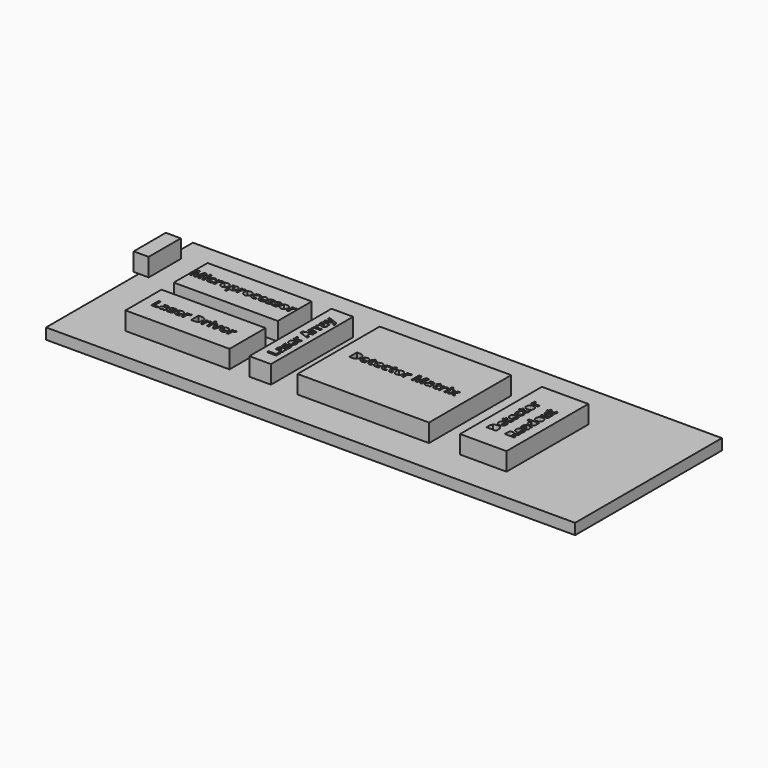
from build123d import *

# Parameters (mm, degrees)
F0_W          = 468.0004864931
F0_H          = 162.3495742679
F1_DEPTH      = 9.652
F3_W          = 19.124776125
F3_H          = 90.8426903188
F4_DEPTH      = 7.112
F4_DEPTH_BACK = 8.89
F3_W_2        = 116.3423849212
F3_W_3        = 1.7658601331
F3_H_2        = 6.4742028383
F3_W_4        = 92.0379832387
F3_H_3        = 39.8432824295
F3_H_4        = 37.4526912346
F3_W_5        = 41.0385876894
F3_H_5        = 90.444251895
F3_W_6        = 13.2810920477
F3_H_6        = 35.5269256979


with BuildPart() as f1:
    # F0 (on Top) → F1 (new body)
    with BuildSketch(Plane.XY):
        with Locations((31.531855464, 13.1481774151)):
            Rectangle(F0_W, F0_H)
    extrude(amount=F1_DEPTH)


with BuildPart() as f4:
    # F3 (on offset) → F4 (new body, two sides)
    with BuildSketch(Plane.XY.offset(22.352)) as f4_sk:
        with Locations((-32.6158255339, 1.7928499728)):
            Rectangle(F3_W, F3_H)
        Polygon((-28.1672623592, -26.0829695182), (-28.1672623592, -31.3119908147), (-36.6333850748, -31.3119908147), (-36.6333850748, -29.5164835021), (-29.6496213377, -29.5164835021), (-29.6496213377, -26.0829695182), align=None, mode=Mode.SUBTRACT)
        with BuildLine():
            Line((-28.1672623592, -19.4067952691), (-28.1672623592, -20.6390061699))
            Line((-28.1672623592, -20.6390061699), (-29.0474130027, -20.9818016837))
            Line((-29.0474130027, -20.9818016837), (-29.0474130027, -21.0281254018))
            add(Edge.make_bspline(
                [(-29.0474130027, -21.0281254018), (-28.4859695396, -21.4728330953), (-28.2682480646, -21.9453350197)],
                knots=[0, 0, 0, 1, 1, 1], degree=2))
            add(Edge.make_bspline(
                [(-28.2682480646, -21.9453350197), (-28.0505265897, -22.417836944), (-28.0505265897, -23.1756929718)],
                knots=[0, 0, 0, 1, 1, 1], degree=2))
            add(Edge.make_bspline(
                [(-28.0505265897, -23.1756929718), (-28.0505265897, -24.1077261795), (-28.5841758219, -24.6432283604)],
                knots=[0, 0, 0, 1, 1, 1], degree=2))
            add(Edge.make_bspline(
                [(-28.5841758219, -24.6432283604), (-29.1178250542, -25.1787305414), (-30.1017408261, -25.1787305414)],
                knots=[0, 0, 0, 1, 1, 1], degree=2))
            add(Edge.make_bspline(
                [(-30.1017408261, -25.1787305414), (-31.1319803161, -25.1787305414), (-31.621158779, -24.4579334881)],
                knots=[0, 0, 0, 1, 1, 1], degree=2))
            add(Edge.make_bspline(
                [(-31.621158779, -24.4579334881), (-32.1103372419, -23.7371364349), (-32.1622198061, -22.284424636)],
                knots=[0, 0, 0, 1, 1, 1], degree=2))
            Line((-32.1622198061, -22.284424636), (-32.1974258319, -21.1596847611))
            Line((-32.1974258319, -21.1596847611), (-32.4809269865, -21.1596847611))
            add(Edge.make_bspline(
                [(-32.4809269865, -21.1596847611), (-33.4648427584, -21.1596847611), (-33.4648427584, -22.1676888664)],
                knots=[0, 0, 0, 1, 1, 1], degree=2))
            add(Edge.make_bspline(
                [(-33.4648427584, -22.1676888664), (-33.4648427584, -22.9440743814), (-32.9960467315, -23.9928433586)],
                knots=[0, 0, 0, 1, 1, 1], degree=2))
            Line((-32.9960467315, -23.9928433586), (-34.1893457091, -24.5765222064))
            add(Edge.make_bspline(
                [(-34.1893457091, -24.5765222064), (-34.7748775056, -23.4591941264), (-34.7748775056, -22.0991297637)],
                knots=[0, 0, 0, 1, 1, 1], degree=2))
            add(Edge.make_bspline(
                [(-34.7748775056, -22.0991297637), (-34.7748775056, -20.7965068114), (-34.206948722, -20.1016510402)],
                knots=[0, 0, 0, 1, 1, 1], degree=2))
            add(Edge.make_bspline(
                [(-34.206948722, -20.1016510402), (-33.6390199384, -19.4067952691), (-32.4809269865, -19.4067952691)],
                knots=[0, 0, 0, 1, 1, 1], degree=2))
            Line((-32.4809269865, -19.4067952691), (-28.1672623592, -19.4067952691))
        make_face(mode=Mode.SUBTRACT)
        with BuildLine():
            add(Edge.make_bspline(
                [(-30.9179647386, -13.2383289701), (-30.570536853, -13.0697106363), (-30.0906231338, -13.0697106363)],
                knots=[0, 0, 0, 1, 1, 1], degree=2))
            add(Edge.make_bspline(
                [(-30.0906231338, -13.0697106363), (-29.0937367208, -13.0697106363), (-28.5721316552, -13.7617869843)],
                knots=[0, 0, 0, 1, 1, 1], degree=2))
            add(Edge.make_bspline(
                [(-28.5721316552, -13.7617869843), (-28.0505265897, -14.4538633324), (-28.0505265897, -15.8324571823)],
                knots=[0, 0, 0, 1, 1, 1], degree=2))
            add(Edge.make_bspline(
                [(-28.0505265897, -15.8324571823), (-28.0505265897, -16.5384306458), (-28.1468799233, -17.0368738523)],
                knots=[0, 0, 0, 1, 1, 1], degree=2))
            add(Edge.make_bspline(
                [(-28.1468799233, -17.0368738523), (-28.2432332569, -17.5353170588), (-28.4285281292, -17.96890706)],
                knots=[0, 0, 0, 1, 1, 1], degree=2))
            Line((-28.4285281292, -17.96890706), (-29.8867987742, -17.96890706))
            add(Edge.make_bspline(
                [(-29.8867987742, -17.96890706), (-29.6551801838, -17.4778756484), (-29.4986060167, -16.8608437236)],
                knots=[0, 0, 0, 1, 1, 1], degree=2))
            add(Edge.make_bspline(
                [(-29.4986060167, -16.8608437236), (-29.3420318496, -16.2438117988), (-29.3420318496, -15.7750157719)],
                knots=[0, 0, 0, 1, 1, 1], degree=2))
            add(Edge.make_bspline(
                [(-29.3420318496, -15.7750157719), (-29.3420318496, -14.8133353846), (-29.8979164666, -14.8133353846)],
                knots=[0, 0, 0, 1, 1, 1], degree=2))
            add(Edge.make_bspline(
                [(-29.8979164666, -14.8133353846), (-30.1072996723, -14.8133353846), (-30.2379325572, -14.9411888465)],
                knots=[0, 0, 0, 1, 1, 1], degree=2))
            add(Edge.make_bspline(
                [(-30.2379325572, -14.9411888465), (-30.3685654422, -15.0690423084), (-30.5334778786, -15.3812641683)],
                knots=[0, 0, 0, 1, 1, 1], degree=2))
            add(Edge.make_bspline(
                [(-30.5334778786, -15.3812641683), (-30.6983903149, -15.6934860281), (-30.9170382642, -16.2141646193)],
                knots=[0, 0, 0, 1, 1, 1], degree=2))
            add(Edge.make_bspline(
                [(-30.9170382642, -16.2141646193), (-31.2301865984, -16.9609029547), (-31.4970112145, -17.3120367377)],
                knots=[0, 0, 0, 1, 1, 1], degree=2))
            add(Edge.make_bspline(
                [(-31.4970112145, -17.3120367377), (-31.7638358307, -17.6631705207), (-32.1084842932, -17.8215976365)],
                knots=[0, 0, 0, 1, 1, 1], degree=2))
            add(Edge.make_bspline(
                [(-32.1084842932, -17.8215976365), (-32.4531327556, -17.9800247523), (-32.9552818596, -17.9800247523)],
                knots=[0, 0, 0, 1, 1, 1], degree=2))
            add(Edge.make_bspline(
                [(-32.9552818596, -17.9800247523), (-33.8187559645, -17.9800247523), (-34.2903314145, -17.3120367377)],
                knots=[0, 0, 0, 1, 1, 1], degree=2))
            add(Edge.make_bspline(
                [(-34.2903314145, -17.3120367377), (-34.7619068646, -16.644048723), (-34.7619068646, -15.4155437196)],
                knots=[0, 0, 0, 1, 1, 1], degree=2))
            add(Edge.make_bspline(
                [(-34.7619068646, -15.4155437196), (-34.7619068646, -14.2463330754), (-34.2523459657, -13.1401226877)],
                knots=[0, 0, 0, 1, 1, 1], degree=2))
            Line((-34.2523459657, -13.1401226877), (-32.979370193, -13.6719189712))
            add(Edge.make_bspline(
                [(-32.979370193, -13.6719189712), (-33.18690045, -14.1592444854), (-33.320312758, -14.5817167943)],
                knots=[0, 0, 0, 1, 1, 1], degree=2))
            add(Edge.make_bspline(
                [(-33.320312758, -14.5817167943), (-33.4537250661, -15.0041891031), (-33.4537250661, -15.4451908992)],
                knots=[0, 0, 0, 1, 1, 1], degree=2))
            add(Edge.make_bspline(
                [(-33.4537250661, -15.4451908992), (-33.4537250661, -16.2271352603), (-33.0312527572, -16.2271352603)],
                knots=[0, 0, 0, 1, 1, 1], degree=2))
            add(Edge.make_bspline(
                [(-33.0312527572, -16.2271352603), (-32.7940753207, -16.2271352603), (-32.6198981407, -15.975134234)],
                knots=[0, 0, 0, 1, 1, 1], degree=2))
            add(Edge.make_bspline(
                [(-32.6198981407, -15.975134234), (-32.4457209608, -15.7231332077), (-32.1047783957, -14.8707767951)],
                knots=[0, 0, 0, 1, 1, 1], degree=2))
            add(Edge.make_bspline(
                [(-32.1047783957, -14.8707767951), (-31.7971889077, -14.1129207673), (-31.5312907659, -13.7599340356)],
                knots=[0, 0, 0, 1, 1, 1], degree=2))
            add(Edge.make_bspline(
                [(-31.5312907659, -13.7599340356), (-31.2653926242, -13.4069473039), (-30.9179647386, -13.2383289701)],
                knots=[0, 0, 0, 1, 1, 1], degree=2))
        make_face(mode=Mode.SUBTRACT)
        with BuildLine():
            add(Edge.make_bspline(
                [(-28.1635564618, -7.4775113901), (-28.0505265897, -8.0037488274), (-28.0505265897, -8.7634578039)],
                knots=[0, 0, 0, 1, 1, 1], degree=2))
            add(Edge.make_bspline(
                [(-28.0505265897, -8.7634578039), (-28.0505265897, -10.3254935774), (-28.9140006946, -11.2056442209)],
                knots=[0, 0, 0, 1, 1, 1], degree=2))
            add(Edge.make_bspline(
                [(-28.9140006946, -11.2056442209), (-29.7774747996, -12.0857948643), (-31.3580400603, -12.0857948643)],
                knots=[0, 0, 0, 1, 1, 1], degree=2))
            add(Edge.make_bspline(
                [(-31.3580400603, -12.0857948643), (-32.9849290392, -12.0857948643), (-33.8734179519, -11.2723503749)],
                knots=[0, 0, 0, 1, 1, 1], degree=2))
            add(Edge.make_bspline(
                [(-33.8734179519, -11.2723503749), (-34.7619068646, -10.4589058855), (-34.7619068646, -9.0228706251)],
                knots=[0, 0, 0, 1, 1, 1], degree=2))
            add(Edge.make_bspline(
                [(-34.7619068646, -9.0228706251), (-34.7619068646, -7.6516885701), (-33.9808889778, -6.8873472218)],
                knots=[0, 0, 0, 1, 1, 1], degree=2))
            add(Edge.make_bspline(
                [(-33.9808889778, -6.8873472218), (-33.199871091, -6.1230058735), (-31.8212772411, -6.1230058735)],
                knots=[0, 0, 0, 1, 1, 1], degree=2))
            Line((-31.8212772411, -6.1230058735), (-30.9633619823, -6.1230058735))
            Line((-30.9633619823, -6.1230058735), (-30.9633619823, -10.2976993466))
            add(Edge.make_bspline(
                [(-30.9633619823, -10.2976993466), (-30.2110648008, -10.268052167), (-29.7885924919, -9.8511387043)],
                knots=[0, 0, 0, 1, 1, 1], degree=2))
            add(Edge.make_bspline(
                [(-29.7885924919, -9.8511387043), (-29.366120183, -9.4342252416), (-29.366120183, -8.6819280601)],
                knots=[0, 0, 0, 1, 1, 1], degree=2))
            add(Edge.make_bspline(
                [(-29.366120183, -8.6819280601), (-29.366120183, -8.0963962636), (-29.4874883244, -7.5757176724)],
                knots=[0, 0, 0, 1, 1, 1], degree=2))
            add(Edge.make_bspline(
                [(-29.4874883244, -7.5757176724), (-29.6088564658, -7.0550390812), (-29.8756810819, -6.488036772)],
                knots=[0, 0, 0, 1, 1, 1], degree=2))
            Line((-29.8756810819, -6.488036772), (-28.5082049243, -6.488036772))
            add(Edge.make_bspline(
                [(-28.5082049243, -6.488036772), (-28.2765863339, -6.9512739527), (-28.1635564618, -7.4775113901)],
                knots=[0, 0, 0, 1, 1, 1], degree=2))
        make_face(mode=Mode.SUBTRACT)
        with BuildLine():
            add(Edge.make_bspline(
                [(-34.4293025688, -2.1882692601), (-34.7619068646, -1.6759289382), (-34.7619068646, -1.0737206032)],
                knots=[0, 0, 0, 1, 1, 1], degree=2))
            add(Edge.make_bspline(
                [(-34.7619068646, -1.0737206032), (-34.7619068646, -0.714248551), (-34.7100243003, -0.4770711144)],
                knots=[0, 0, 0, 1, 1, 1], degree=2))
            Line((-34.7100243003, -0.4770711144), (-33.0553410906, -0.6104834225))
            add(Edge.make_bspline(
                [(-33.0553410906, -0.6104834225), (-33.112782501, -0.8254254743), (-33.112782501, -1.1311620136)],
                knots=[0, 0, 0, 1, 1, 1], degree=2))
            add(Edge.make_bspline(
                [(-33.112782501, -1.1311620136), (-33.112782501, -1.9761066314), (-32.6782660255, -2.4486085557)],
                knots=[0, 0, 0, 1, 1, 1], degree=2))
            add(Edge.make_bspline(
                [(-32.6782660255, -2.4486085557), (-32.2437495499, -2.9211104801), (-31.4618051888, -2.9211104801)],
                knots=[0, 0, 0, 1, 1, 1], degree=2))
            Line((-31.4618051888, -2.9211104801), (-28.1672623592, -2.9211104801))
            Line((-28.1672623592, -2.9211104801), (-28.1672623592, -4.6869706132))
            Line((-28.1672623592, -4.6869706132), (-34.6414651976, -4.6869706132))
            Line((-34.6414651976, -4.6869706132), (-34.6414651976, -3.3491416351))
            Line((-34.6414651976, -3.3491416351), (-33.5519313484, -3.0878758652))
            Line((-33.5519313484, -3.0878758652), (-33.5519313484, -3.0026402239))
            add(Edge.make_bspline(
                [(-33.5519313484, -3.0026402239), (-34.096698273, -2.7006095821), (-34.4293025688, -2.1882692601)],
                knots=[0, 0, 0, 1, 1, 1], degree=2))
        make_face(mode=Mode.SUBTRACT)
        Polygon((-28.1672623592, 11.0352993019), (-28.1672623592, 9.100820835), (-30.1832705699, 8.4874948077), (-30.1832705699, 5.4004822351), (-28.1672623592, 4.7871562078), (-28.1672623592, 2.8526777409), (-36.6685911006, 5.8414840312), (-36.6685911006, 8.0353753193), align=None, mode=Mode.SUBTRACT)
        with BuildLine():
            add(Edge.make_bspline(
                [(-34.4293025688, 14.4604750165), (-34.7619068646, 14.9728153384), (-34.7619068646, 15.5750236734)],
                knots=[0, 0, 0, 1, 1, 1], degree=2))
            add(Edge.make_bspline(
                [(-34.7619068646, 15.5750236734), (-34.7619068646, 15.9344957257), (-34.7100243003, 16.1716731622)],
                knots=[0, 0, 0, 1, 1, 1], degree=2))
            Line((-34.7100243003, 16.1716731622), (-33.0553410906, 16.0382608541))
            add(Edge.make_bspline(
                [(-33.0553410906, 16.0382608541), (-33.112782501, 15.8233188023), (-33.112782501, 15.517582263)],
                knots=[0, 0, 0, 1, 1, 1], degree=2))
            add(Edge.make_bspline(
                [(-33.112782501, 15.517582263), (-33.112782501, 14.6726376453), (-32.6782660255, 14.2001357209)],
                knots=[0, 0, 0, 1, 1, 1], degree=2))
            add(Edge.make_bspline(
                [(-32.6782660255, 14.2001357209), (-32.2437495499, 13.7276337965), (-31.4618051888, 13.7276337965)],
                knots=[0, 0, 0, 1, 1, 1], degree=2))
            Line((-31.4618051888, 13.7276337965), (-28.1672623592, 13.7276337965))
            Line((-28.1672623592, 13.7276337965), (-28.1672623592, 11.9617736634))
            Line((-28.1672623592, 11.9617736634), (-34.6414651976, 11.9617736634))
            Line((-34.6414651976, 11.9617736634), (-34.6414651976, 13.2996026415))
            Line((-34.6414651976, 13.2996026415), (-33.5519313484, 13.5608684114))
            Line((-33.5519313484, 13.5608684114), (-33.5519313484, 13.6461040527))
            add(Edge.make_bspline(
                [(-33.5519313484, 13.6461040527), (-34.096698273, 13.9481346945), (-34.4293025688, 14.4604750165)],
                knots=[0, 0, 0, 1, 1, 1], degree=2))
        make_face(mode=Mode.SUBTRACT)
        with BuildLine():
            add(Edge.make_bspline(
                [(-34.4293025688, 19.8451440057), (-34.7619068646, 20.3574843276), (-34.7619068646, 20.9596926626)],
                knots=[0, 0, 0, 1, 1, 1], degree=2))
            add(Edge.make_bspline(
                [(-34.7619068646, 20.9596926626), (-34.7619068646, 21.3191647148), (-34.7100243003, 21.5563421514)],
                knots=[0, 0, 0, 1, 1, 1], degree=2))
            Line((-34.7100243003, 21.5563421514), (-33.0553410906, 21.4229298433))
            add(Edge.make_bspline(
                [(-33.0553410906, 21.4229298433), (-33.112782501, 21.2079877915), (-33.112782501, 20.9022512522)],
                knots=[0, 0, 0, 1, 1, 1], degree=2))
            add(Edge.make_bspline(
                [(-33.112782501, 20.9022512522), (-33.112782501, 20.0573066344), (-32.6782660255, 19.5848047101)],
                knots=[0, 0, 0, 1, 1, 1], degree=2))
            add(Edge.make_bspline(
                [(-32.6782660255, 19.5848047101), (-32.2437495499, 19.1123027857), (-31.4618051888, 19.1123027857)],
                knots=[0, 0, 0, 1, 1, 1], degree=2))
            Line((-31.4618051888, 19.1123027857), (-28.1672623592, 19.1123027857))
            Line((-28.1672623592, 19.1123027857), (-28.1672623592, 17.3464426526))
            Line((-28.1672623592, 17.3464426526), (-34.6414651976, 17.3464426526))
            Line((-34.6414651976, 17.3464426526), (-34.6414651976, 18.6842716307))
            Line((-34.6414651976, 18.6842716307), (-33.5519313484, 18.9455374006))
            Line((-33.5519313484, 18.9455374006), (-33.5519313484, 19.0307730419))
            add(Edge.make_bspline(
                [(-33.5519313484, 19.0307730419), (-34.096698273, 19.3328036837), (-34.4293025688, 19.8451440057)],
                knots=[0, 0, 0, 1, 1, 1], degree=2))
        make_face(mode=Mode.SUBTRACT)
        with BuildLine():
            Line((-28.1672623592, 28.0750157591), (-28.1672623592, 26.8428048583))
            Line((-28.1672623592, 26.8428048583), (-29.0474130027, 26.5000093445))
            Line((-29.0474130027, 26.5000093445), (-29.0474130027, 26.4536856264))
            add(Edge.make_bspline(
                [(-29.0474130027, 26.4536856264), (-28.4859695396, 26.0089779329), (-28.2682480646, 25.5364760085)],
                knots=[0, 0, 0, 1, 1, 1], degree=2))
            add(Edge.make_bspline(
                [(-28.2682480646, 25.5364760085), (-28.0505265897, 25.0639740841), (-28.0505265897, 24.3061180564)],
                knots=[0, 0, 0, 1, 1, 1], degree=2))
            add(Edge.make_bspline(
                [(-28.0505265897, 24.3061180564), (-28.0505265897, 23.3740848487), (-28.5841758219, 22.8385826677)],
                knots=[0, 0, 0, 1, 1, 1], degree=2))
            add(Edge.make_bspline(
                [(-28.5841758219, 22.8385826677), (-29.1178250542, 22.3030804868), (-30.1017408261, 22.3030804868)],
                knots=[0, 0, 0, 1, 1, 1], degree=2))
            add(Edge.make_bspline(
                [(-30.1017408261, 22.3030804868), (-31.1319803161, 22.3030804868), (-31.621158779, 23.02387754)],
                knots=[0, 0, 0, 1, 1, 1], degree=2))
            add(Edge.make_bspline(
                [(-31.621158779, 23.02387754), (-32.1103372419, 23.7446745933), (-32.1622198061, 25.1973863922)],
                knots=[0, 0, 0, 1, 1, 1], degree=2))
            Line((-32.1622198061, 25.1973863922), (-32.1974258319, 26.3221262671))
            Line((-32.1974258319, 26.3221262671), (-32.4809269865, 26.3221262671))
            add(Edge.make_bspline(
                [(-32.4809269865, 26.3221262671), (-33.4648427584, 26.3221262671), (-33.4648427584, 25.3141221617)],
                knots=[0, 0, 0, 1, 1, 1], degree=2))
            add(Edge.make_bspline(
                [(-33.4648427584, 25.3141221617), (-33.4648427584, 24.5377366468), (-32.9960467315, 23.4889676695)],
                knots=[0, 0, 0, 1, 1, 1], degree=2))
            Line((-32.9960467315, 23.4889676695), (-34.1893457091, 22.9052888218))
            add(Edge.make_bspline(
                [(-34.1893457091, 22.9052888218), (-34.7748775056, 24.0226169018), (-34.7748775056, 25.3826812645)],
                knots=[0, 0, 0, 1, 1, 1], degree=2))
            add(Edge.make_bspline(
                [(-34.7748775056, 25.3826812645), (-34.7748775056, 26.6853042168), (-34.206948722, 27.3801599879)],
                knots=[0, 0, 0, 1, 1, 1], degree=2))
            add(Edge.make_bspline(
                [(-34.206948722, 27.3801599879), (-33.6390199384, 28.0750157591), (-32.4809269865, 28.0750157591)],
                knots=[0, 0, 0, 1, 1, 1], degree=2))
            Line((-32.4809269865, 28.0750157591), (-28.1672623592, 28.0750157591))
        make_face(mode=Mode.SUBTRACT)
        with BuildLine():
            Line((-28.2135860773, 31.5400298712), (-34.6414651976, 28.9681370436))
            Line((-34.6414651976, 28.9681370436), (-34.6414651976, 30.9026155105))
            Line((-34.6414651976, 30.9026155105), (-30.998568008, 32.1237087189))
            add(Edge.make_bspline(
                [(-30.998568008, 32.1237087189), (-30.5242131349, 32.2812093604), (-29.8756810819, 32.3386507708)],
                knots=[0, 0, 0, 1, 1, 1], degree=2))
            Line((-29.8756810819, 32.3386507708), (-29.8756810819, 32.3738567966))
            add(Edge.make_bspline(
                [(-29.8756810819, 32.3738567966), (-30.4723305707, 32.4368570531), (-30.998568008, 32.6221519254)],
                knots=[0, 0, 0, 1, 1, 1], degree=2))
            Line((-30.998568008, 32.6221519254), (-34.6414651976, 33.8210097493))
            Line((-34.6414651976, 33.8210097493), (-34.6414651976, 35.7147233442))
            Line((-34.6414651976, 35.7147233442), (-27.33899428, 32.9760651315))
            add(Edge.make_bspline(
                [(-27.33899428, 32.9760651315), (-26.3254313285, 32.598063592), (-25.8214292758, 31.9004283978)],
                knots=[0, 0, 0, 1, 1, 1], degree=2))
            add(Edge.make_bspline(
                [(-25.8214292758, 31.9004283978), (-25.3174272232, 31.2027932036), (-25.3174272232, 30.2707599959)],
                knots=[0, 0, 0, 1, 1, 1], degree=2))
            add(Edge.make_bspline(
                [(-25.3174272232, 30.2707599959), (-25.3174272232, 29.8130816613), (-25.4174864542, 29.3739328139)],
                knots=[0, 0, 0, 1, 1, 1], degree=2))
            Line((-25.4174864542, 29.3739328139), (-26.8183156888, 29.3739328139))
            add(Edge.make_bspline(
                [(-26.8183156888, 29.3739328139), (-26.7423447912, 29.6926399943), (-26.7423447912, 30.0687885851)],
                knots=[0, 0, 0, 1, 1, 1], degree=2))
            add(Edge.make_bspline(
                [(-26.7423447912, 30.0687885851), (-26.7423447912, 30.537584612), (-27.0295518433, 30.8877919207)],
                knots=[0, 0, 0, 1, 1, 1], degree=2))
            add(Edge.make_bspline(
                [(-27.0295518433, 30.8877919207), (-27.3167588953, 31.2379992293), (-27.8948788969, 31.434411794)],
                knots=[0, 0, 0, 1, 1, 1], degree=2))
            Line((-27.8948788969, 31.434411794), (-28.2135860773, 31.5400298712))
        make_face(mode=Mode.SUBTRACT)
    extrude(amount=F4_DEPTH)
    extrude(f4_sk.sketch, amount=-F4_DEPTH_BACK)


with BuildPart() as f4b:
    # F3 (on offset) → F4, piece 2 (new body, two sides)
    with BuildSketch(Plane.XY.offset(22.352)) as f4_2_sk:
        with Locations((58.6252936191, 1.7928499728)):
            Rectangle(F3_W_2, F3_H)
        with BuildLine():
            add(Edge.make_bspline(
                [(25.2443428277, -1.3248665976), (24.7181053904, -1.4378964697), (23.9583964139, -1.4378964697)],
                knots=[0, 0, 0, 1, 1, 1], degree=2))
            add(Edge.make_bspline(
                [(23.9583964139, -1.4378964697), (22.3963606404, -1.4378964697), (21.516209997, -0.5744223648)],
                knots=[0, 0, 0, 1, 1, 1], degree=2))
            add(Edge.make_bspline(
                [(21.516209997, -0.5744223648), (20.6360593535, 0.2890517402), (20.6360593535, 1.8696170009)],
                knots=[0, 0, 0, 1, 1, 1], degree=2))
            add(Edge.make_bspline(
                [(20.6360593535, 1.8696170009), (20.6360593535, 3.4965059798), (21.4495038429, 4.3849948925)],
                knots=[0, 0, 0, 1, 1, 1], degree=2))
            add(Edge.make_bspline(
                [(21.4495038429, 4.3849948925), (22.2629483324, 5.2734838052), (23.6989835927, 5.2734838052)],
                knots=[0, 0, 0, 1, 1, 1], degree=2))
            add(Edge.make_bspline(
                [(23.6989835927, 5.2734838052), (25.0701656478, 5.2734838052), (25.834506996, 4.4924659184)],
                knots=[0, 0, 0, 1, 1, 1], degree=2))
            add(Edge.make_bspline(
                [(25.834506996, 4.4924659184), (26.5988483443, 3.7114480316), (26.5988483443, 2.3328541817)],
                knots=[0, 0, 0, 1, 1, 1], degree=2))
            Line((26.5988483443, 2.3328541817), (26.5988483443, 1.4749389229))
            Line((26.5988483443, 1.4749389229), (22.4241548713, 1.4749389229))
            add(Edge.make_bspline(
                [(22.4241548713, 1.4749389229), (22.4538020508, 0.7226417414), (22.8707155135, 0.3001694325)],
                knots=[0, 0, 0, 1, 1, 1], degree=2))
            add(Edge.make_bspline(
                [(22.8707155135, 0.3001694325), (23.2876289762, -0.1223028764), (24.0399261578, -0.1223028764)],
                knots=[0, 0, 0, 1, 1, 1], degree=2))
            add(Edge.make_bspline(
                [(24.0399261578, -0.1223028764), (24.6254579542, -0.1223028764), (25.1461365454, -0.000934735)],
                knots=[0, 0, 0, 1, 1, 1], degree=2))
            add(Edge.make_bspline(
                [(25.1461365454, -0.000934735), (25.6668151366, 0.1204334064), (26.2338174459, 0.3872580225)],
                knots=[0, 0, 0, 1, 1, 1], degree=2))
            Line((26.2338174459, 0.3872580225), (26.2338174459, -0.9802181351))
            add(Edge.make_bspline(
                [(26.2338174459, -0.9802181351), (25.7705802651, -1.2118367255), (25.2443428277, -1.3248665976)],
                knots=[0, 0, 0, 1, 1, 1], degree=2))
        make_face(mode=Mode.SUBTRACT)
        with BuildLine():
            add(Edge.make_bspline(
                [(18.2661379367, 6.0507957945), (19.4131131963, 4.9566295735), (19.4131131963, 2.9925039271)],
                knots=[0, 0, 0, 1, 1, 1], degree=2))
            add(Edge.make_bspline(
                [(19.4131131963, 2.9925039271), (19.4131131963, 0.9023777675), (18.2225936417, -0.2093914663)],
                knots=[0, 0, 0, 1, 1, 1], degree=2))
            add(Edge.make_bspline(
                [(18.2225936417, -0.2093914663), (17.0320740872, -1.3211607002), (14.7863002348, -1.3211607002)],
                knots=[0, 0, 0, 1, 1, 1], degree=2))
            Line((14.7863002348, -1.3211607002), (12.3885845872, -1.3211607002))
            Line((12.3885845872, -1.3211607002), (12.3885845872, 7.1449620154))
            Line((12.3885845872, 7.1449620154), (15.0457130561, 7.1449620154))
            add(Edge.make_bspline(
                [(15.0457130561, 7.1449620154), (17.1191626772, 7.1449620154), (18.2661379367, 6.0507957945)],
                knots=[0, 0, 0, 1, 1, 1], degree=2))
        make_face(mode=Mode.SUBTRACT)
        with BuildLine():
            add(Edge.make_bspline(
                [(37.3978335022, -1.3248665976), (36.8715960649, -1.4378964697), (36.1118870884, -1.4378964697)],
                knots=[0, 0, 0, 1, 1, 1], degree=2))
            add(Edge.make_bspline(
                [(36.1118870884, -1.4378964697), (34.5498513149, -1.4378964697), (33.6697006715, -0.5744223648)],
                knots=[0, 0, 0, 1, 1, 1], degree=2))
            add(Edge.make_bspline(
                [(33.6697006715, -0.5744223648), (32.789550028, 0.2890517402), (32.789550028, 1.8696170009)],
                knots=[0, 0, 0, 1, 1, 1], degree=2))
            add(Edge.make_bspline(
                [(32.789550028, 1.8696170009), (32.789550028, 3.4965059798), (33.6029945174, 4.3849948925)],
                knots=[0, 0, 0, 1, 1, 1], degree=2))
            add(Edge.make_bspline(
                [(33.6029945174, 4.3849948925), (34.4164390068, 5.2734838052), (35.8524742672, 5.2734838052)],
                knots=[0, 0, 0, 1, 1, 1], degree=2))
            add(Edge.make_bspline(
                [(35.8524742672, 5.2734838052), (37.2236563223, 5.2734838052), (37.9879976705, 4.4924659184)],
                knots=[0, 0, 0, 1, 1, 1], degree=2))
            add(Edge.make_bspline(
                [(37.9879976705, 4.4924659184), (38.7523390188, 3.7114480316), (38.7523390188, 2.3328541817)],
                knots=[0, 0, 0, 1, 1, 1], degree=2))
            Line((38.7523390188, 2.3328541817), (38.7523390188, 1.4749389229))
            Line((38.7523390188, 1.4749389229), (34.5776455457, 1.4749389229))
            add(Edge.make_bspline(
                [(34.5776455457, 1.4749389229), (34.6072927253, 0.7226417414), (35.024206188, 0.3001694325)],
                knots=[0, 0, 0, 1, 1, 1], degree=2))
            add(Edge.make_bspline(
                [(35.024206188, 0.3001694325), (35.4411196507, -0.1223028764), (36.1934168322, -0.1223028764)],
                knots=[0, 0, 0, 1, 1, 1], degree=2))
            add(Edge.make_bspline(
                [(36.1934168322, -0.1223028764), (36.7789486287, -0.1223028764), (37.2996272199, -0.000934735)],
                knots=[0, 0, 0, 1, 1, 1], degree=2))
            add(Edge.make_bspline(
                [(37.2996272199, -0.000934735), (37.8203058111, 0.1204334064), (38.3873081203, 0.3872580225)],
                knots=[0, 0, 0, 1, 1, 1], degree=2))
            Line((38.3873081203, 0.3872580225), (38.3873081203, -0.9802181351))
            add(Edge.make_bspline(
                [(38.3873081203, -0.9802181351), (37.9240709396, -1.2118367255), (37.3978335022, -1.3248665976)],
                knots=[0, 0, 0, 1, 1, 1], degree=2))
        make_face(mode=Mode.SUBTRACT)
        with BuildLine():
            add(Edge.make_bspline(
                [(30.2028336106, 0.1500805859), (30.4140697651, -0.0296554402), (30.762424125, -0.0296554402)],
                knots=[0, 0, 0, 1, 1, 1], degree=2))
            add(Edge.make_bspline(
                [(30.762424125, -0.0296554402), (31.2256613057, -0.0296554402), (31.8741933588, 0.1723159706)],
                knots=[0, 0, 0, 1, 1, 1], degree=2))
            Line((31.8741933588, 0.1723159706), (31.8741933588, -1.141424674))
            add(Edge.make_bspline(
                [(31.8741933588, -1.141424674), (31.2145436134, -1.4378964697), (30.2528632261, -1.4378964697)],
                knots=[0, 0, 0, 1, 1, 1], degree=2))
            add(Edge.make_bspline(
                [(30.2528632261, -1.4378964697), (29.1929765566, -1.4378964697), (28.7093569398, -0.9014678144)],
                knots=[0, 0, 0, 1, 1, 1], degree=2))
            add(Edge.make_bspline(
                [(28.7093569398, -0.9014678144), (28.2257373231, -0.3650391591), (28.2257373231, 0.7059652028)],
                knots=[0, 0, 0, 1, 1, 1], degree=2))
            Line((28.2257373231, 0.7059652028), (28.2257373231, 3.8263308525))
            Line((28.2257373231, 3.8263308525), (27.3807927054, 3.8263308525))
            Line((27.3807927054, 3.8263308525), (27.3807927054, 4.5730691879))
            Line((27.3807927054, 4.5730691879), (28.353590785, 5.1641598305))
            Line((28.353590785, 5.1641598305), (28.8631516839, 6.5316359881))
            Line((28.8631516839, 6.5316359881), (29.9915974562, 6.5316359881))
            Line((29.9915974562, 6.5316359881), (29.9915974562, 5.1530421382))
            Line((29.9915974562, 5.1530421382), (31.8037813073, 5.1530421382))
            Line((31.8037813073, 5.1530421382), (31.8037813073, 3.8263308525))
            Line((31.8037813073, 3.8263308525), (29.9915974562, 3.8263308525))
            Line((29.9915974562, 3.8263308525), (29.9915974562, 0.7059652028))
            add(Edge.make_bspline(
                [(29.9915974562, 0.7059652028), (29.9915974562, 0.3298166121), (30.2028336106, 0.1500805859)],
                knots=[0, 0, 0, 1, 1, 1], degree=2))
        make_face(mode=Mode.SUBTRACT)
        with BuildLine():
            add(Edge.make_bspline(
                [(43.9202130074, -1.3332048669), (43.4829171087, -1.4378964697), (42.8177085172, -1.4378964697)],
                knots=[0, 0, 0, 1, 1, 1], degree=2))
            add(Edge.make_bspline(
                [(42.8177085172, -1.4378964697), (39.7955491499, -1.4378964697), (39.7955491499, 1.8807346933)],
                knots=[0, 0, 0, 1, 1, 1], degree=2))
            add(Edge.make_bspline(
                [(39.7955491499, 1.8807346933), (39.7955491499, 3.5317120055), (40.6173319085, 4.4025979053)],
                knots=[0, 0, 0, 1, 1, 1], degree=2))
            add(Edge.make_bspline(
                [(40.6173319085, 4.4025979053), (41.4391146672, 5.2734838052), (42.9733562099, 5.2734838052)],
                knots=[0, 0, 0, 1, 1, 1], degree=2))
            add(Edge.make_bspline(
                [(42.9733562099, 5.2734838052), (44.0962431361, 5.2734838052), (44.9893644206, 4.8343349578)],
                knots=[0, 0, 0, 1, 1, 1], degree=2))
            Line((44.9893644206, 4.8343349578), (44.4668328807, 3.4668588002))
            add(Edge.make_bspline(
                [(44.4668328807, 3.4668588002), (44.049919418, 3.635477134), (43.6913738401, 3.7429481599)],
                knots=[0, 0, 0, 1, 1, 1], degree=2))
            add(Edge.make_bspline(
                [(43.6913738401, 3.7429481599), (43.3328282622, 3.8504191859), (42.9733562099, 3.8504191859)],
                knots=[0, 0, 0, 1, 1, 1], degree=2))
            add(Edge.make_bspline(
                [(42.9733562099, 3.8504191859), (41.5947623599, 3.8504191859), (41.5947623599, 1.8918523856)],
                knots=[0, 0, 0, 1, 1, 1], degree=2))
            add(Edge.make_bspline(
                [(41.5947623599, 1.8918523856), (41.5947623599, -0.0074200555), (42.9733562099, -0.0074200555)],
                knots=[0, 0, 0, 1, 1, 1], degree=2))
            add(Edge.make_bspline(
                [(42.9733562099, -0.0074200555), (43.4829171087, -0.0074200555), (43.9174335843, 0.1287716756)],
                knots=[0, 0, 0, 1, 1, 1], degree=2))
            add(Edge.make_bspline(
                [(43.9174335843, 0.1287716756), (44.3519500598, 0.2649634068), (44.785540061, 0.5558763563)],
                knots=[0, 0, 0, 1, 1, 1], degree=2))
            Line((44.785540061, 0.5558763563), (44.785540061, -0.9561298017))
            add(Edge.make_bspline(
                [(44.785540061, -0.9561298017), (44.357508906, -1.228513264), (43.9202130074, -1.3332048669)],
                knots=[0, 0, 0, 1, 1, 1], degree=2))
        make_face(mode=Mode.SUBTRACT)
        with BuildLine():
            add(Edge.make_bspline(
                [(48.4543785327, 0.1500805859), (48.6656146871, -0.0296554402), (49.013969047, -0.0296554402)],
                knots=[0, 0, 0, 1, 1, 1], degree=2))
            add(Edge.make_bspline(
                [(49.013969047, -0.0296554402), (49.4772062278, -0.0296554402), (50.1257382809, 0.1723159706)],
                knots=[0, 0, 0, 1, 1, 1], degree=2))
            Line((50.1257382809, 0.1723159706), (50.1257382809, -1.141424674))
            add(Edge.make_bspline(
                [(50.1257382809, -1.141424674), (49.4660885355, -1.4378964697), (48.5044081482, -1.4378964697)],
                knots=[0, 0, 0, 1, 1, 1], degree=2))
            add(Edge.make_bspline(
                [(48.5044081482, -1.4378964697), (47.4445214786, -1.4378964697), (46.9609018619, -0.9014678144)],
                knots=[0, 0, 0, 1, 1, 1], degree=2))
            add(Edge.make_bspline(
                [(46.9609018619, -0.9014678144), (46.4772822452, -0.3650391591), (46.4772822452, 0.7059652028)],
                knots=[0, 0, 0, 1, 1, 1], degree=2))
            Line((46.4772822452, 0.7059652028), (46.4772822452, 3.8263308525))
            Line((46.4772822452, 3.8263308525), (45.6323376275, 3.8263308525))
            Line((45.6323376275, 3.8263308525), (45.6323376275, 4.5730691879))
            Line((45.6323376275, 4.5730691879), (46.6051357071, 5.1641598305))
            Line((46.6051357071, 5.1641598305), (47.1146966059, 6.5316359881))
            Line((47.1146966059, 6.5316359881), (48.2431423782, 6.5316359881))
            Line((48.2431423782, 6.5316359881), (48.2431423782, 5.1530421382))
            Line((48.2431423782, 5.1530421382), (50.0553262294, 5.1530421382))
            Line((50.0553262294, 5.1530421382), (50.0553262294, 3.8263308525))
            Line((50.0553262294, 3.8263308525), (48.2431423782, 3.8263308525))
            Line((48.2431423782, 3.8263308525), (48.2431423782, 0.7059652028))
            add(Edge.make_bspline(
                [(48.2431423782, 0.7059652028), (48.2431423782, 0.3298166121), (48.4543785327, 0.1500805859)],
                knots=[0, 0, 0, 1, 1, 1], degree=2))
        make_face(mode=Mode.SUBTRACT)
        with BuildLine():
            add(Edge.make_bspline(
                [(56.9353248381, 3.7049627111), (57.317032275, 2.946180209), (57.317032275, 1.9270584113)],
                knots=[0, 0, 0, 1, 1, 1], degree=2))
            add(Edge.make_bspline(
                [(57.317032275, 1.9270584113), (57.317032275, 0.3464931506), (56.4832053497, -0.5457016596)],
                knots=[0, 0, 0, 1, 1, 1], degree=2))
            add(Edge.make_bspline(
                [(56.4832053497, -0.5457016596), (55.6493784243, -1.4378964697), (54.1614605997, -1.4378964697)],
                knots=[0, 0, 0, 1, 1, 1], degree=2))
            add(Edge.make_bspline(
                [(54.1614605997, -1.4378964697), (53.229427392, -1.4378964697), (52.516968608, -1.0293212763)],
                knots=[0, 0, 0, 1, 1, 1], degree=2))
            add(Edge.make_bspline(
                [(52.516968608, -1.0293212763), (51.8045098239, -0.6207460829), (51.422802387, 0.1435952654)],
                knots=[0, 0, 0, 1, 1, 1], degree=2))
            add(Edge.make_bspline(
                [(51.422802387, 0.1435952654), (51.0410949501, 0.9079366137), (51.0410949501, 1.9270584113)],
                knots=[0, 0, 0, 1, 1, 1], degree=2))
            add(Edge.make_bspline(
                [(51.0410949501, 1.9270584113), (51.0410949501, 3.5131825183), (51.8684365549, 4.3933331617)],
                knots=[0, 0, 0, 1, 1, 1], degree=2))
            add(Edge.make_bspline(
                [(51.8684365549, 4.3933331617), (52.6957781597, 5.2734838052), (54.1966666254, 5.2734838052)],
                knots=[0, 0, 0, 1, 1, 1], degree=2))
            add(Edge.make_bspline(
                [(54.1966666254, 5.2734838052), (55.1286998331, 5.2734838052), (55.8411586171, 4.8686145092)],
                knots=[0, 0, 0, 1, 1, 1], degree=2))
            add(Edge.make_bspline(
                [(55.8411586171, 4.8686145092), (56.5536174011, 4.4637452132), (56.9353248381, 3.7049627111)],
                knots=[0, 0, 0, 1, 1, 1], degree=2))
        make_face(mode=Mode.SUBTRACT)
        with BuildLine():
            add(Edge.make_bspline(
                [(61.2758572218, 4.9408795094), (61.7881975437, 5.2734838052), (62.3904058787, 5.2734838052)],
                knots=[0, 0, 0, 1, 1, 1], degree=2))
            add(Edge.make_bspline(
                [(62.3904058787, 5.2734838052), (62.749877931, 5.2734838052), (62.9870553676, 5.2216012409)],
                knots=[0, 0, 0, 1, 1, 1], degree=2))
            Line((62.9870553676, 5.2216012409), (62.8536430595, 3.5669180312))
            add(Edge.make_bspline(
                [(62.8536430595, 3.5669180312), (62.6387010076, 3.6243594416), (62.3329644683, 3.6243594416)],
                knots=[0, 0, 0, 1, 1, 1], degree=2))
            add(Edge.make_bspline(
                [(62.3329644683, 3.6243594416), (61.4880198506, 3.6243594416), (61.0155179262, 3.1898429661)],
                knots=[0, 0, 0, 1, 1, 1], degree=2))
            add(Edge.make_bspline(
                [(61.0155179262, 3.1898429661), (60.5430160019, 2.7553264905), (60.5430160019, 1.9733821294)],
                knots=[0, 0, 0, 1, 1, 1], degree=2))
            Line((60.5430160019, 1.9733821294), (60.5430160019, -1.3211607002))
            Line((60.5430160019, -1.3211607002), (58.7771558688, -1.3211607002))
            Line((58.7771558688, -1.3211607002), (58.7771558688, 5.1530421382))
            Line((58.7771558688, 5.1530421382), (60.1149848468, 5.1530421382))
            Line((60.1149848468, 5.1530421382), (60.3762506168, 4.063508289))
            Line((60.3762506168, 4.063508289), (60.461486258, 4.063508289))
            add(Edge.make_bspline(
                [(60.461486258, 4.063508289), (60.7635168999, 4.6082752136), (61.2758572218, 4.9408795094)],
                knots=[0, 0, 0, 1, 1, 1], degree=2))
        make_face(mode=Mode.SUBTRACT)
        with BuildLine():
            Line((72.6112710351, -1.3211607002), (70.965852569, -1.3211607002))
            Line((70.965852569, -1.3211607002), (68.9276089737, 5.3198075232))
            Line((68.9276089737, 5.3198075232), (68.8757264094, 5.3198075232))
            add(Edge.make_bspline(
                [(68.8757264094, 5.3198075232), (68.9869033328, 3.2945345689), (68.9869033328, 2.6163553363)],
                knots=[0, 0, 0, 1, 1, 1], degree=2))
            Line((68.9869033328, 2.6163553363), (68.9869033328, -1.3211607002))
            Line((68.9869033328, -1.3211607002), (67.3822497386, -1.3211607002))
            Line((67.3822497386, -1.3211607002), (67.3822497386, 7.1449620154))
            Line((67.3822497386, 7.1449620154), (69.8262891043, 7.1449620154))
            Line((69.8262891043, 7.1449620154), (71.829326674, 0.6707591771))
            Line((71.829326674, 0.6707591771), (71.8645326997, 0.6707591771))
            Line((71.8645326997, 0.6707591771), (73.989864885, 7.1449620154))
            Line((73.989864885, 7.1449620154), (76.432051302, 7.1449620154))
            Line((76.432051302, 7.1449620154), (76.432051302, -1.3211607002))
            Line((76.432051302, -1.3211607002), (74.7588386051, -1.3211607002))
            Line((74.7588386051, -1.3211607002), (74.7588386051, 2.6867673878))
            add(Edge.make_bspline(
                [(74.7588386051, 2.6867673878), (74.7588386051, 2.9702685424), (74.7681033487, 3.340858287)],
                knots=[0, 0, 0, 1, 1, 1], degree=2))
            add(Edge.make_bspline(
                [(74.7681033487, 3.340858287), (74.7773680923, 3.7114480316), (74.8459271951, 5.3086898309)],
                knots=[0, 0, 0, 1, 1, 1], degree=2))
            Line((74.8459271951, 5.3086898309), (74.7940446308, 5.3086898309))
            Line((74.7940446308, 5.3086898309), (72.6112710351, -1.3211607002))
        make_face(mode=Mode.SUBTRACT)
        with BuildLine():
            Line((83.7678752966, -1.3211607002), (82.5356643957, -1.3211607002))
            Line((82.5356643957, -1.3211607002), (82.192868882, -0.4410100567))
            Line((82.192868882, -0.4410100567), (82.1465451639, -0.4410100567))
            add(Edge.make_bspline(
                [(82.1465451639, -0.4410100567), (81.7018374704, -1.0024535198), (81.229335546, -1.2201749948)],
                knots=[0, 0, 0, 1, 1, 1], degree=2))
            add(Edge.make_bspline(
                [(81.229335546, -1.2201749948), (80.7568336216, -1.4378964697), (79.9989775939, -1.4378964697)],
                knots=[0, 0, 0, 1, 1, 1], degree=2))
            add(Edge.make_bspline(
                [(79.9989775939, -1.4378964697), (79.0669443862, -1.4378964697), (78.5314422052, -0.9042472375)],
                knots=[0, 0, 0, 1, 1, 1], degree=2))
            add(Edge.make_bspline(
                [(78.5314422052, -0.9042472375), (77.9959400243, -0.3705980052), (77.9959400243, 0.6133177667)],
                knots=[0, 0, 0, 1, 1, 1], degree=2))
            add(Edge.make_bspline(
                [(77.9959400243, 0.6133177667), (77.9959400243, 1.6435572567), (78.7167370775, 2.1327357196)],
                knots=[0, 0, 0, 1, 1, 1], degree=2))
            add(Edge.make_bspline(
                [(78.7167370775, 2.1327357196), (79.4375341308, 2.6219141825), (80.8902459297, 2.6737967467)],
                knots=[0, 0, 0, 1, 1, 1], degree=2))
            Line((80.8902459297, 2.6737967467), (82.0149858046, 2.7090027725))
            Line((82.0149858046, 2.7090027725), (82.0149858046, 2.9925039271))
            add(Edge.make_bspline(
                [(82.0149858046, 2.9925039271), (82.0149858046, 3.976419699), (81.0069816992, 3.976419699)],
                knots=[0, 0, 0, 1, 1, 1], degree=2))
            add(Edge.make_bspline(
                [(81.0069816992, 3.976419699), (80.2305961843, 3.976419699), (79.181827207, 3.5076236721)],
                knots=[0, 0, 0, 1, 1, 1], degree=2))
            Line((79.181827207, 3.5076236721), (78.5981483593, 4.7009226497))
            add(Edge.make_bspline(
                [(78.5981483593, 4.7009226497), (79.7154764393, 5.2864544462), (81.075540802, 5.2864544462)],
                knots=[0, 0, 0, 1, 1, 1], degree=2))
            add(Edge.make_bspline(
                [(81.075540802, 5.2864544462), (82.3781637543, 5.2864544462), (83.0730195254, 4.7185256626)],
                knots=[0, 0, 0, 1, 1, 1], degree=2))
            add(Edge.make_bspline(
                [(83.0730195254, 4.7185256626), (83.7678752966, 4.150596879), (83.7678752966, 2.9925039271)],
                knots=[0, 0, 0, 1, 1, 1], degree=2))
            Line((83.7678752966, 2.9925039271), (83.7678752966, -1.3211607002))
        make_face(mode=Mode.SUBTRACT)
        with BuildLine():
            add(Edge.make_bspline(
                [(87.7554209486, 0.1500805859), (87.966657103, -0.0296554402), (88.3150114629, -0.0296554402)],
                knots=[0, 0, 0, 1, 1, 1], degree=2))
            add(Edge.make_bspline(
                [(88.3150114629, -0.0296554402), (88.7782486437, -0.0296554402), (89.4267806968, 0.1723159706)],
                knots=[0, 0, 0, 1, 1, 1], degree=2))
            Line((89.4267806968, 0.1723159706), (89.4267806968, -1.141424674))
            add(Edge.make_bspline(
                [(89.4267806968, -1.141424674), (88.7671309514, -1.4378964697), (87.8054505641, -1.4378964697)],
                knots=[0, 0, 0, 1, 1, 1], degree=2))
            add(Edge.make_bspline(
                [(87.8054505641, -1.4378964697), (86.7455638945, -1.4378964697), (86.2619442778, -0.9014678144)],
                knots=[0, 0, 0, 1, 1, 1], degree=2))
            add(Edge.make_bspline(
                [(86.2619442778, -0.9014678144), (85.7783246611, -0.3650391591), (85.7783246611, 0.7059652028)],
                knots=[0, 0, 0, 1, 1, 1], degree=2))
            Line((85.7783246611, 0.7059652028), (85.7783246611, 3.8263308525))
            Line((85.7783246611, 3.8263308525), (84.9333800434, 3.8263308525))
            Line((84.9333800434, 3.8263308525), (84.9333800434, 4.5730691879))
            Line((84.9333800434, 4.5730691879), (85.906178123, 5.1641598305))
            Line((85.906178123, 5.1641598305), (86.4157390218, 6.5316359881))
            Line((86.4157390218, 6.5316359881), (87.5441847941, 6.5316359881))
            Line((87.5441847941, 6.5316359881), (87.5441847941, 5.1530421382))
            Line((87.5441847941, 5.1530421382), (89.3563686453, 5.1530421382))
            Line((89.3563686453, 5.1530421382), (89.3563686453, 3.8263308525))
            Line((89.3563686453, 3.8263308525), (87.5441847941, 3.8263308525))
            Line((87.5441847941, 3.8263308525), (87.5441847941, 0.7059652028))
            add(Edge.make_bspline(
                [(87.5441847941, 0.7059652028), (87.5441847941, 0.3298166121), (87.7554209486, 0.1500805859)],
                knots=[0, 0, 0, 1, 1, 1], degree=2))
        make_face(mode=Mode.SUBTRACT)
        with Locations((97.002561551, 1.915940719)):
            Rectangle(F3_W_3, F3_H_2, mode=Mode.SUBTRACT)
        with BuildLine():
            add(Edge.make_bspline(
                [(93.2336638483, 4.9408795094), (93.7460041702, 5.2734838052), (94.3482125052, 5.2734838052)],
                knots=[0, 0, 0, 1, 1, 1], degree=2))
            add(Edge.make_bspline(
                [(94.3482125052, 5.2734838052), (94.7076845575, 5.2734838052), (94.944861994, 5.2216012409)],
                knots=[0, 0, 0, 1, 1, 1], degree=2))
            Line((94.944861994, 5.2216012409), (94.8114496859, 3.5669180312))
            add(Edge.make_bspline(
                [(94.8114496859, 3.5669180312), (94.5965076341, 3.6243594416), (94.2907710948, 3.6243594416)],
                knots=[0, 0, 0, 1, 1, 1], degree=2))
            add(Edge.make_bspline(
                [(94.2907710948, 3.6243594416), (93.4458264771, 3.6243594416), (92.9733245527, 3.1898429661)],
                knots=[0, 0, 0, 1, 1, 1], degree=2))
            add(Edge.make_bspline(
                [(92.9733245527, 3.1898429661), (92.5008226283, 2.7553264905), (92.5008226283, 1.9733821294)],
                knots=[0, 0, 0, 1, 1, 1], degree=2))
            Line((92.5008226283, 1.9733821294), (92.5008226283, -1.3211607002))
            Line((92.5008226283, -1.3211607002), (90.7349624952, -1.3211607002))
            Line((90.7349624952, -1.3211607002), (90.7349624952, 5.1530421382))
            Line((90.7349624952, 5.1530421382), (92.0727914733, 5.1530421382))
            Line((92.0727914733, 5.1530421382), (92.3340572432, 4.063508289))
            Line((92.3340572432, 4.063508289), (92.4192928845, 4.063508289))
            add(Edge.make_bspline(
                [(92.4192928845, 4.063508289), (92.7213235263, 4.6082752136), (93.2336638483, 4.9408795094)],
                knots=[0, 0, 0, 1, 1, 1], degree=2))
        make_face(mode=Mode.SUBTRACT)
        Polygon((98.8694073894, -1.3211607002), (101.0651516262, 1.9844998217), (98.9805843128, 5.1530421382), (100.9836218824, 5.1530421382), (102.2399211167, 3.0907102094), (103.5073380432, 5.1530421382), (105.5122285616, 5.1530421382), (103.4035729147, 1.9844998217), (105.6104348439, -1.3211607002), (103.5999854794, -1.3211607002), (102.2399211167, 0.8968189213), (100.8742979078, -1.3211607002), align=None, mode=Mode.SUBTRACT)
        with BuildLine():
            add(Edge.make_bspline(
                [(97.005340974, 5.957221884), (96.0436605868, 5.957221884), (96.0436605868, 6.8262548351)],
                knots=[0, 0, 0, 1, 1, 1], degree=2))
            add(Edge.make_bspline(
                [(96.0436605868, 6.8262548351), (96.0436605868, 7.68972894), (97.005340974, 7.68972894)],
                knots=[0, 0, 0, 1, 1, 1], degree=2))
            add(Edge.make_bspline(
                [(97.005340974, 7.68972894), (97.9670213613, 7.68972894), (97.9670213613, 6.8262548351)],
                knots=[0, 0, 0, 1, 1, 1], degree=2))
            add(Edge.make_bspline(
                [(97.9670213613, 6.8262548351), (97.9670213613, 6.4149002186), (97.7270645017, 6.1860610513)],
                knots=[0, 0, 0, 1, 1, 1], degree=2))
            add(Edge.make_bspline(
                [(97.7270645017, 6.1860610513), (97.487107642, 5.957221884), (97.005340974, 5.957221884)],
                knots=[0, 0, 0, 1, 1, 1], degree=2))
        make_face(mode=Mode.SUBTRACT)
    extrude(amount=F4_DEPTH)
    extrude(f4_2_sk.sketch, amount=-F4_DEPTH_BACK)


with BuildPart() as f4c:
    # F3 (on offset) → F4, piece 3 (new body, two sides)
    with BuildSketch(Plane.XY.offset(22.352)) as f4_3_sk:
        with Locations((-105.7282499969, -23.7068539718)):
            Rectangle(F3_W_4, F3_H_3)
        with BuildLine():
            Line((-130.7522730979, -26.6215372831), (-131.9844839988, -26.6215372831))
            Line((-131.9844839988, -26.6215372831), (-132.3272795125, -25.7413866396))
            Line((-132.3272795125, -25.7413866396), (-132.3736032306, -25.7413866396))
            add(Edge.make_bspline(
                [(-132.3736032306, -25.7413866396), (-132.8183109241, -26.3028301027), (-133.2908128485, -26.5205515777)],
                knots=[0, 0, 0, 1, 1, 1], degree=2))
            add(Edge.make_bspline(
                [(-133.2908128485, -26.5205515777), (-133.7633147729, -26.7382730526), (-134.5211708006, -26.7382730526)],
                knots=[0, 0, 0, 1, 1, 1], degree=2))
            add(Edge.make_bspline(
                [(-134.5211708006, -26.7382730526), (-135.4532040083, -26.7382730526), (-135.9887061893, -26.2046238204)],
                knots=[0, 0, 0, 1, 1, 1], degree=2))
            add(Edge.make_bspline(
                [(-135.9887061893, -26.2046238204), (-136.5242083702, -25.6709745881), (-136.5242083702, -24.6870588162)],
                knots=[0, 0, 0, 1, 1, 1], degree=2))
            add(Edge.make_bspline(
                [(-136.5242083702, -24.6870588162), (-136.5242083702, -23.6568193262), (-135.803411317, -23.1676408633)],
                knots=[0, 0, 0, 1, 1, 1], degree=2))
            add(Edge.make_bspline(
                [(-135.803411317, -23.1676408633), (-135.0826142637, -22.6784624004), (-133.6299024648, -22.6265798362)],
                knots=[0, 0, 0, 1, 1, 1], degree=2))
            Line((-133.6299024648, -22.6265798362), (-132.50516259, -22.5913738104))
            Line((-132.50516259, -22.5913738104), (-132.50516259, -22.3078726558))
            add(Edge.make_bspline(
                [(-132.50516259, -22.3078726558), (-132.50516259, -21.3239568839), (-133.5131666953, -21.3239568839)],
                knots=[0, 0, 0, 1, 1, 1], degree=2))
            add(Edge.make_bspline(
                [(-133.5131666953, -21.3239568839), (-134.2895522102, -21.3239568839), (-135.3383211875, -21.7927529108)],
                knots=[0, 0, 0, 1, 1, 1], degree=2))
            Line((-135.3383211875, -21.7927529108), (-135.9220000353, -20.5994539331))
            add(Edge.make_bspline(
                [(-135.9220000353, -20.5994539331), (-134.8046719553, -20.0139221367), (-133.4446075925, -20.0139221367)],
                knots=[0, 0, 0, 1, 1, 1], degree=2))
            add(Edge.make_bspline(
                [(-133.4446075925, -20.0139221367), (-132.1419846402, -20.0139221367), (-131.4471288691, -20.5818509203)],
                knots=[0, 0, 0, 1, 1, 1], degree=2))
            add(Edge.make_bspline(
                [(-131.4471288691, -20.5818509203), (-130.7522730979, -21.1497797039), (-130.7522730979, -22.3078726558)],
                knots=[0, 0, 0, 1, 1, 1], degree=2))
            Line((-130.7522730979, -22.3078726558), (-130.7522730979, -26.6215372831))
        make_face(mode=Mode.SUBTRACT)
        with BuildLine():
            add(Edge.make_bspline(
                [(-124.5838067989, -23.8708349037), (-124.4151884651, -24.2182627893), (-124.4151884651, -24.6981765085)],
                knots=[0, 0, 0, 1, 1, 1], degree=2))
            add(Edge.make_bspline(
                [(-124.4151884651, -24.6981765085), (-124.4151884651, -25.6950629215), (-125.1072648132, -26.2166679871)],
                knots=[0, 0, 0, 1, 1, 1], degree=2))
            add(Edge.make_bspline(
                [(-125.1072648132, -26.2166679871), (-125.7993411612, -26.7382730526), (-127.1779350112, -26.7382730526)],
                knots=[0, 0, 0, 1, 1, 1], degree=2))
            add(Edge.make_bspline(
                [(-127.1779350112, -26.7382730526), (-127.8839084747, -26.7382730526), (-128.3823516812, -26.641919719)],
                knots=[0, 0, 0, 1, 1, 1], degree=2))
            add(Edge.make_bspline(
                [(-128.3823516812, -26.641919719), (-128.8807948877, -26.5455663854), (-129.3143848889, -26.3602715131)],
                knots=[0, 0, 0, 1, 1, 1], degree=2))
            Line((-129.3143848889, -26.3602715131), (-129.3143848889, -24.9020008681))
            add(Edge.make_bspline(
                [(-129.3143848889, -24.9020008681), (-128.8233534772, -25.1336194585), (-128.2063215525, -25.2901936256)],
                knots=[0, 0, 0, 1, 1, 1], degree=2))
            add(Edge.make_bspline(
                [(-128.2063215525, -25.2901936256), (-127.5892896277, -25.4467677926), (-127.1204936008, -25.4467677926)],
                knots=[0, 0, 0, 1, 1, 1], degree=2))
            add(Edge.make_bspline(
                [(-127.1204936008, -25.4467677926), (-126.1588132135, -25.4467677926), (-126.1588132135, -24.8908831757)],
                knots=[0, 0, 0, 1, 1, 1], degree=2))
            add(Edge.make_bspline(
                [(-126.1588132135, -24.8908831757), (-126.1588132135, -24.68149997), (-126.2866666754, -24.5508670851)],
                knots=[0, 0, 0, 1, 1, 1], degree=2))
            add(Edge.make_bspline(
                [(-126.2866666754, -24.5508670851), (-126.4145201373, -24.4202342001), (-126.7267419971, -24.2553217637)],
                knots=[0, 0, 0, 1, 1, 1], degree=2))
            add(Edge.make_bspline(
                [(-126.7267419971, -24.2553217637), (-127.038963857, -24.0904093274), (-127.5596424481, -23.8717613781)],
                knots=[0, 0, 0, 1, 1, 1], degree=2))
            add(Edge.make_bspline(
                [(-127.5596424481, -23.8717613781), (-128.3063807835, -23.5586130439), (-128.6575145665, -23.2917884277)],
                knots=[0, 0, 0, 1, 1, 1], degree=2))
            add(Edge.make_bspline(
                [(-128.6575145665, -23.2917884277), (-129.0086483496, -23.0249638116), (-129.1670754654, -22.6803153491)],
                knots=[0, 0, 0, 1, 1, 1], degree=2))
            add(Edge.make_bspline(
                [(-129.1670754654, -22.6803153491), (-129.3255025812, -22.3356668866), (-129.3255025812, -21.8335177827)],
                knots=[0, 0, 0, 1, 1, 1], degree=2))
            add(Edge.make_bspline(
                [(-129.3255025812, -21.8335177827), (-129.3255025812, -20.9700436778), (-128.6575145665, -20.4984682277)],
                knots=[0, 0, 0, 1, 1, 1], degree=2))
            add(Edge.make_bspline(
                [(-128.6575145665, -20.4984682277), (-127.9895265519, -20.0268927777), (-126.7610215485, -20.0268927777)],
                knots=[0, 0, 0, 1, 1, 1], degree=2))
            add(Edge.make_bspline(
                [(-126.7610215485, -20.0268927777), (-125.5918109042, -20.0268927777), (-124.4856005166, -20.5364536766)],
                knots=[0, 0, 0, 1, 1, 1], degree=2))
            Line((-124.4856005166, -20.5364536766), (-125.0173968001, -21.8094294493))
            add(Edge.make_bspline(
                [(-125.0173968001, -21.8094294493), (-125.5047223143, -21.6018991923), (-125.9271946231, -21.4684868843)],
                knots=[0, 0, 0, 1, 1, 1], degree=2))
            add(Edge.make_bspline(
                [(-125.9271946231, -21.4684868843), (-126.349666932, -21.3350745762), (-126.7906687281, -21.3350745762)],
                knots=[0, 0, 0, 1, 1, 1], degree=2))
            add(Edge.make_bspline(
                [(-126.7906687281, -21.3350745762), (-127.5726130892, -21.3350745762), (-127.5726130892, -21.7575468851)],
                knots=[0, 0, 0, 1, 1, 1], degree=2))
            add(Edge.make_bspline(
                [(-127.5726130892, -21.7575468851), (-127.5726130892, -21.9947243216), (-127.3206120629, -22.1689015016)],
                knots=[0, 0, 0, 1, 1, 1], degree=2))
            add(Edge.make_bspline(
                [(-127.3206120629, -22.1689015016), (-127.0686110365, -22.3430786815), (-126.2162546239, -22.6840212466)],
                knots=[0, 0, 0, 1, 1, 1], degree=2))
            add(Edge.make_bspline(
                [(-126.2162546239, -22.6840212466), (-125.4583985962, -22.9916107346), (-125.1054118644, -23.2575088764)],
                knots=[0, 0, 0, 1, 1, 1], degree=2))
            add(Edge.make_bspline(
                [(-125.1054118644, -23.2575088764), (-124.7524251327, -23.5234070181), (-124.5838067989, -23.8708349037)],
                knots=[0, 0, 0, 1, 1, 1], degree=2))
        make_face(mode=Mode.SUBTRACT)
        with BuildLine():
            add(Edge.make_bspline(
                [(-118.8229892189, -26.6252431805), (-119.3492266563, -26.7382730526), (-120.1089356327, -26.7382730526)],
                knots=[0, 0, 0, 1, 1, 1], degree=2))
            add(Edge.make_bspline(
                [(-120.1089356327, -26.7382730526), (-121.6709714063, -26.7382730526), (-122.5511220497, -25.8747989477)],
                knots=[0, 0, 0, 1, 1, 1], degree=2))
            add(Edge.make_bspline(
                [(-122.5511220497, -25.8747989477), (-123.4312726932, -25.0113248427), (-123.4312726932, -23.430759582)],
                knots=[0, 0, 0, 1, 1, 1], degree=2))
            add(Edge.make_bspline(
                [(-123.4312726932, -23.430759582), (-123.4312726932, -21.8038706031), (-122.6178282038, -20.9153816904)],
                knots=[0, 0, 0, 1, 1, 1], degree=2))
            add(Edge.make_bspline(
                [(-122.6178282038, -20.9153816904), (-121.8043837143, -20.0268927777), (-120.368348454, -20.0268927777)],
                knots=[0, 0, 0, 1, 1, 1], degree=2))
            add(Edge.make_bspline(
                [(-120.368348454, -20.0268927777), (-118.9971663989, -20.0268927777), (-118.2328250507, -20.8079106645)],
                knots=[0, 0, 0, 1, 1, 1], degree=2))
            add(Edge.make_bspline(
                [(-118.2328250507, -20.8079106645), (-117.4684837024, -21.5889285513), (-117.4684837024, -22.9675224012)],
                knots=[0, 0, 0, 1, 1, 1], degree=2))
            Line((-117.4684837024, -22.9675224012), (-117.4684837024, -23.82543766))
            Line((-117.4684837024, -23.82543766), (-121.6431771754, -23.82543766))
            add(Edge.make_bspline(
                [(-121.6431771754, -23.82543766), (-121.6135299959, -24.5777348415), (-121.1966165332, -25.0002071504)],
                knots=[0, 0, 0, 1, 1, 1], degree=2))
            add(Edge.make_bspline(
                [(-121.1966165332, -25.0002071504), (-120.7797030705, -25.4226794592), (-120.0274058889, -25.4226794592)],
                knots=[0, 0, 0, 1, 1, 1], degree=2))
            add(Edge.make_bspline(
                [(-120.0274058889, -25.4226794592), (-119.4418740924, -25.4226794592), (-118.9211955013, -25.3013113179)],
                knots=[0, 0, 0, 1, 1, 1], degree=2))
            add(Edge.make_bspline(
                [(-118.9211955013, -25.3013113179), (-118.4005169101, -25.1799431765), (-117.8335146008, -24.9131185604)],
                knots=[0, 0, 0, 1, 1, 1], degree=2))
            Line((-117.8335146008, -24.9131185604), (-117.8335146008, -26.280594718))
            add(Edge.make_bspline(
                [(-117.8335146008, -26.280594718), (-118.2967517816, -26.5122133084), (-118.8229892189, -26.6252431805)],
                knots=[0, 0, 0, 1, 1, 1], degree=2))
        make_face(mode=Mode.SUBTRACT)
        Polygon((-137.4284473471, -26.6215372831), (-142.6574686435, -26.6215372831), (-142.6574686435, -18.1554145674), (-140.8619613309, -18.1554145674), (-140.8619613309, -25.1391783046), (-137.4284473471, -25.1391783046), align=None, mode=Mode.SUBTRACT)
        with BuildLine():
            add(Edge.make_bspline(
                [(-113.533747089, -20.3594970735), (-113.0214067671, -20.0268927777), (-112.4191984321, -20.0268927777)],
                knots=[0, 0, 0, 1, 1, 1], degree=2))
            add(Edge.make_bspline(
                [(-112.4191984321, -20.0268927777), (-112.0597263798, -20.0268927777), (-111.8225489433, -20.078775342)],
                knots=[0, 0, 0, 1, 1, 1], degree=2))
            Line((-111.8225489433, -20.078775342), (-111.9559612513, -21.7334585517))
            add(Edge.make_bspline(
                [(-111.9559612513, -21.7334585517), (-112.1709033032, -21.6760171412), (-112.4766398425, -21.6760171412)],
                knots=[0, 0, 0, 1, 1, 1], degree=2))
            add(Edge.make_bspline(
                [(-112.4766398425, -21.6760171412), (-113.3215844602, -21.6760171412), (-113.7940863846, -22.1105336168)],
                knots=[0, 0, 0, 1, 1, 1], degree=2))
            add(Edge.make_bspline(
                [(-113.7940863846, -22.1105336168), (-114.266588309, -22.5450500924), (-114.266588309, -23.3269944535)],
                knots=[0, 0, 0, 1, 1, 1], degree=2))
            Line((-114.266588309, -23.3269944535), (-114.266588309, -26.6215372831))
            Line((-114.266588309, -26.6215372831), (-116.032448442, -26.6215372831))
            Line((-116.032448442, -26.6215372831), (-116.032448442, -20.1473344447))
            Line((-116.032448442, -20.1473344447), (-114.694619464, -20.1473344447))
            Line((-114.694619464, -20.1473344447), (-114.433353694, -21.2368682939))
            Line((-114.433353694, -21.2368682939), (-114.3481180528, -21.2368682939))
            add(Edge.make_bspline(
                [(-114.3481180528, -21.2368682939), (-114.0460874109, -20.6921013693), (-113.533747089, -20.3594970735)],
                knots=[0, 0, 0, 1, 1, 1], degree=2))
        make_face(mode=Mode.SUBTRACT)
        with Locations((-92.5194556209, -23.3844358639)):
            Rectangle(F3_W_3, F3_H_2, mode=Mode.SUBTRACT)
        with BuildLine():
            Line((-86.4315925913, -26.6215372831), (-88.2437764424, -26.6215372831))
            Line((-88.2437764424, -26.6215372831), (-90.7100511928, -20.1473344447))
            Line((-90.7100511928, -20.1473344447), (-88.8626613159, -20.1473344447))
            Line((-88.8626613159, -20.1473344447), (-87.6119209279, -23.8365553523))
            add(Edge.make_bspline(
                [(-87.6119209279, -23.8365553523), (-87.4043906709, -24.5369699696), (-87.3506551579, -25.1614136893)],
                knots=[0, 0, 0, 1, 1, 1], degree=2))
            Line((-87.3506551579, -25.1614136893), (-87.3173020809, -25.1614136893))
            add(Edge.make_bspline(
                [(-87.3173020809, -25.1614136893), (-87.2876549014, -24.6055290724), (-87.056036311, -23.8365553523)],
                knots=[0, 0, 0, 1, 1, 1], degree=2))
            Line((-87.056036311, -23.8365553523), (-85.8108547691, -20.1473344447))
            Line((-85.8108547691, -20.1473344447), (-83.9634648922, -20.1473344447))
            Line((-83.9634648922, -20.1473344447), (-86.4315925913, -26.6215372831))
        make_face(mode=Mode.SUBTRACT)
        with BuildLine():
            add(Edge.make_bspline(
                [(-78.8215321857, -26.6252431805), (-79.3477696231, -26.7382730526), (-80.1074785995, -26.7382730526)],
                knots=[0, 0, 0, 1, 1, 1], degree=2))
            add(Edge.make_bspline(
                [(-80.1074785995, -26.7382730526), (-81.6695143731, -26.7382730526), (-82.5496650165, -25.8747989477)],
                knots=[0, 0, 0, 1, 1, 1], degree=2))
            add(Edge.make_bspline(
                [(-82.5496650165, -25.8747989477), (-83.42981566, -25.0113248427), (-83.42981566, -23.430759582)],
                knots=[0, 0, 0, 1, 1, 1], degree=2))
            add(Edge.make_bspline(
                [(-83.42981566, -23.430759582), (-83.42981566, -21.8038706031), (-82.6163711705, -20.9153816904)],
                knots=[0, 0, 0, 1, 1, 1], degree=2))
            add(Edge.make_bspline(
                [(-82.6163711705, -20.9153816904), (-81.8029266811, -20.0268927777), (-80.3668914208, -20.0268927777)],
                knots=[0, 0, 0, 1, 1, 1], degree=2))
            add(Edge.make_bspline(
                [(-80.3668914208, -20.0268927777), (-78.9957093657, -20.0268927777), (-78.2313680174, -20.8079106645)],
                knots=[0, 0, 0, 1, 1, 1], degree=2))
            add(Edge.make_bspline(
                [(-78.2313680174, -20.8079106645), (-77.4670266692, -21.5889285513), (-77.4670266692, -22.9675224012)],
                knots=[0, 0, 0, 1, 1, 1], degree=2))
            Line((-77.4670266692, -22.9675224012), (-77.4670266692, -23.82543766))
            Line((-77.4670266692, -23.82543766), (-81.6417201422, -23.82543766))
            add(Edge.make_bspline(
                [(-81.6417201422, -23.82543766), (-81.6120729626, -24.5777348415), (-81.1951595, -25.0002071504)],
                knots=[0, 0, 0, 1, 1, 1], degree=2))
            add(Edge.make_bspline(
                [(-81.1951595, -25.0002071504), (-80.7782460373, -25.4226794592), (-80.0259488557, -25.4226794592)],
                knots=[0, 0, 0, 1, 1, 1], degree=2))
            add(Edge.make_bspline(
                [(-80.0259488557, -25.4226794592), (-79.4404170592, -25.4226794592), (-78.9197384681, -25.3013113179)],
                knots=[0, 0, 0, 1, 1, 1], degree=2))
            add(Edge.make_bspline(
                [(-78.9197384681, -25.3013113179), (-78.3990598769, -25.1799431765), (-77.8320575676, -24.9131185604)],
                knots=[0, 0, 0, 1, 1, 1], degree=2))
            Line((-77.8320575676, -24.9131185604), (-77.8320575676, -26.280594718))
            add(Edge.make_bspline(
                [(-77.8320575676, -26.280594718), (-78.2952947484, -26.5122133084), (-78.8215321857, -26.6252431805)],
                knots=[0, 0, 0, 1, 1, 1], degree=2))
        make_face(mode=Mode.SUBTRACT)
        with BuildLine():
            add(Edge.make_bspline(
                [(-101.5498012227, -19.2495807884), (-100.4028259631, -20.3437470094), (-100.4028259631, -22.3078726558)],
                knots=[0, 0, 0, 1, 1, 1], degree=2))
            add(Edge.make_bspline(
                [(-100.4028259631, -22.3078726558), (-100.4028259631, -24.3979988154), (-101.5933455177, -25.5097680492)],
                knots=[0, 0, 0, 1, 1, 1], degree=2))
            add(Edge.make_bspline(
                [(-101.5933455177, -25.5097680492), (-102.7838650722, -26.6215372831), (-105.0296389246, -26.6215372831)],
                knots=[0, 0, 0, 1, 1, 1], degree=2))
            Line((-105.0296389246, -26.6215372831), (-107.4273545722, -26.6215372831))
            Line((-107.4273545722, -26.6215372831), (-107.4273545722, -18.1554145674))
            Line((-107.4273545722, -18.1554145674), (-104.7702261033, -18.1554145674))
            add(Edge.make_bspline(
                [(-104.7702261033, -18.1554145674), (-102.6967764822, -18.1554145674), (-101.5498012227, -19.2495807884)],
                knots=[0, 0, 0, 1, 1, 1], degree=2))
        make_face(mode=Mode.SUBTRACT)
        with BuildLine():
            add(Edge.make_bspline(
                [(-96.2883533236, -20.3594970735), (-95.7760130016, -20.0268927777), (-95.1738046667, -20.0268927777)],
                knots=[0, 0, 0, 1, 1, 1], degree=2))
            add(Edge.make_bspline(
                [(-95.1738046667, -20.0268927777), (-94.8143326144, -20.0268927777), (-94.5771551778, -20.078775342)],
                knots=[0, 0, 0, 1, 1, 1], degree=2))
            Line((-94.5771551778, -20.078775342), (-94.7105674859, -21.7334585517))
            add(Edge.make_bspline(
                [(-94.7105674859, -21.7334585517), (-94.9255095378, -21.6760171412), (-95.2312460771, -21.6760171412)],
                knots=[0, 0, 0, 1, 1, 1], degree=2))
            add(Edge.make_bspline(
                [(-95.2312460771, -21.6760171412), (-96.0761906948, -21.6760171412), (-96.5486926192, -22.1105336168)],
                knots=[0, 0, 0, 1, 1, 1], degree=2))
            add(Edge.make_bspline(
                [(-96.5486926192, -22.1105336168), (-97.0211945435, -22.5450500924), (-97.0211945435, -23.3269944535)],
                knots=[0, 0, 0, 1, 1, 1], degree=2))
            Line((-97.0211945435, -23.3269944535), (-97.0211945435, -26.6215372831))
            Line((-97.0211945435, -26.6215372831), (-98.7870546766, -26.6215372831))
            Line((-98.7870546766, -26.6215372831), (-98.7870546766, -20.1473344447))
            Line((-98.7870546766, -20.1473344447), (-97.4492256986, -20.1473344447))
            Line((-97.4492256986, -20.1473344447), (-97.1879599286, -21.2368682939))
            Line((-97.1879599286, -21.2368682939), (-97.1027242873, -21.2368682939))
            add(Edge.make_bspline(
                [(-97.1027242873, -21.2368682939), (-96.8006936455, -20.6921013693), (-96.2883533236, -20.3594970735)],
                knots=[0, 0, 0, 1, 1, 1], degree=2))
        make_face(mode=Mode.SUBTRACT)
        with BuildLine():
            add(Edge.make_bspline(
                [(-92.5166761978, -19.3431546989), (-93.4783565851, -19.3431546989), (-93.4783565851, -18.4741217478)],
                knots=[0, 0, 0, 1, 1, 1], degree=2))
            add(Edge.make_bspline(
                [(-93.4783565851, -18.4741217478), (-93.4783565851, -17.6106476429), (-92.5166761978, -17.6106476429)],
                knots=[0, 0, 0, 1, 1, 1], degree=2))
            add(Edge.make_bspline(
                [(-92.5166761978, -17.6106476429), (-91.5549958105, -17.6106476429), (-91.5549958105, -18.4741217478)],
                knots=[0, 0, 0, 1, 1, 1], degree=2))
            add(Edge.make_bspline(
                [(-91.5549958105, -18.4741217478), (-91.5549958105, -18.8854763643), (-91.7949526702, -19.1143155316)],
                knots=[0, 0, 0, 1, 1, 1], degree=2))
            add(Edge.make_bspline(
                [(-91.7949526702, -19.1143155316), (-92.0349095298, -19.3431546989), (-92.5166761978, -19.3431546989)],
                knots=[0, 0, 0, 1, 1, 1], degree=2))
        make_face(mode=Mode.SUBTRACT)
        with BuildLine():
            add(Edge.make_bspline(
                [(-73.5322900558, -20.3594970735), (-73.0199497339, -20.0268927777), (-72.4177413989, -20.0268927777)],
                knots=[0, 0, 0, 1, 1, 1], degree=2))
            add(Edge.make_bspline(
                [(-72.4177413989, -20.0268927777), (-72.0582693466, -20.0268927777), (-71.82109191, -20.078775342)],
                knots=[0, 0, 0, 1, 1, 1], degree=2))
            Line((-71.82109191, -20.078775342), (-71.9545042181, -21.7334585517))
            add(Edge.make_bspline(
                [(-71.9545042181, -21.7334585517), (-72.16944627, -21.6760171412), (-72.4751828093, -21.6760171412)],
                knots=[0, 0, 0, 1, 1, 1], degree=2))
            add(Edge.make_bspline(
                [(-72.4751828093, -21.6760171412), (-73.320127427, -21.6760171412), (-73.7926293514, -22.1105336168)],
                knots=[0, 0, 0, 1, 1, 1], degree=2))
            add(Edge.make_bspline(
                [(-73.7926293514, -22.1105336168), (-74.2651312758, -22.5450500924), (-74.2651312758, -23.3269944535)],
                knots=[0, 0, 0, 1, 1, 1], degree=2))
            Line((-74.2651312758, -23.3269944535), (-74.2651312758, -26.6215372831))
            Line((-74.2651312758, -26.6215372831), (-76.0309914088, -26.6215372831))
            Line((-76.0309914088, -26.6215372831), (-76.0309914088, -20.1473344447))
            Line((-76.0309914088, -20.1473344447), (-74.6931624308, -20.1473344447))
            Line((-74.6931624308, -20.1473344447), (-74.4318966608, -21.2368682939))
            Line((-74.4318966608, -21.2368682939), (-74.3466610196, -21.2368682939))
            add(Edge.make_bspline(
                [(-74.3466610196, -21.2368682939), (-74.0446303777, -20.6921013693), (-73.5322900558, -20.3594970735)],
                knots=[0, 0, 0, 1, 1, 1], degree=2))
        make_face(mode=Mode.SUBTRACT)
    extrude(amount=F4_DEPTH)
    extrude(f4_3_sk.sketch, amount=-F4_DEPTH_BACK)


with BuildPart() as f4d:
    # F3 (on offset) → F4, piece 4 (new body, two sides)
    with BuildSketch(Plane.XY.offset(22.352)) as f4_4_sk:
        with Locations((-105.7282499969, 28.4878495149)):
            Rectangle(F3_W_4, F3_H_4)
        with BuildLine():
            Line((-145.452774804, 25.7724896073), (-147.0981932701, 25.7724896073))
            Line((-147.0981932701, 25.7724896073), (-149.1364368655, 32.4134578307))
            Line((-149.1364368655, 32.4134578307), (-149.1883194297, 32.4134578307))
            add(Edge.make_bspline(
                [(-149.1883194297, 32.4134578307), (-149.0771425063, 30.3881848765), (-149.0771425063, 29.7100056438)],
                knots=[0, 0, 0, 1, 1, 1], degree=2))
            Line((-149.0771425063, 29.7100056438), (-149.0771425063, 25.7724896073))
            Line((-149.0771425063, 25.7724896073), (-150.6817961005, 25.7724896073))
            Line((-150.6817961005, 25.7724896073), (-150.6817961005, 34.238612323))
            Line((-150.6817961005, 34.238612323), (-148.2377567348, 34.238612323))
            Line((-148.2377567348, 34.238612323), (-146.2347191652, 27.7644094846))
            Line((-146.2347191652, 27.7644094846), (-146.1995131394, 27.7644094846))
            Line((-146.1995131394, 27.7644094846), (-144.0741809541, 34.238612323))
            Line((-144.0741809541, 34.238612323), (-141.6319945371, 34.238612323))
            Line((-141.6319945371, 34.238612323), (-141.6319945371, 25.7724896073))
            Line((-141.6319945371, 25.7724896073), (-143.305207234, 25.7724896073))
            Line((-143.305207234, 25.7724896073), (-143.305207234, 29.7804176953))
            add(Edge.make_bspline(
                [(-143.305207234, 29.7804176953), (-143.305207234, 30.0639188499), (-143.2959424904, 30.4345085945)],
                knots=[0, 0, 0, 1, 1, 1], degree=2))
            add(Edge.make_bspline(
                [(-143.2959424904, 30.4345085945), (-143.2866777468, 30.8050983391), (-143.218118644, 32.4023401384)],
                knots=[0, 0, 0, 1, 1, 1], degree=2))
            Line((-143.218118644, 32.4023401384), (-143.2700012083, 32.4023401384))
            Line((-143.2700012083, 32.4023401384), (-145.452774804, 25.7724896073))
        make_face(mode=Mode.SUBTRACT)
        with Locations((-138.7571445933, 29.0095910265)):
            Rectangle(F3_W_3, F3_H_2, mode=Mode.SUBTRACT)
        with BuildLine():
            add(Edge.make_bspline(
                [(-132.2894270755, 25.7604454406), (-132.7267229741, 25.6557538378), (-133.3919315657, 25.6557538378)],
                knots=[0, 0, 0, 1, 1, 1], degree=2))
            add(Edge.make_bspline(
                [(-133.3919315657, 25.6557538378), (-136.414090933, 25.6557538378), (-136.414090933, 28.9743850008)],
                knots=[0, 0, 0, 1, 1, 1], degree=2))
            add(Edge.make_bspline(
                [(-136.414090933, 28.9743850008), (-136.414090933, 30.625362313), (-135.5923081743, 31.4962482128)],
                knots=[0, 0, 0, 1, 1, 1], degree=2))
            add(Edge.make_bspline(
                [(-135.5923081743, 31.4962482128), (-134.7705254157, 32.3671341127), (-133.236283873, 32.3671341127)],
                knots=[0, 0, 0, 1, 1, 1], degree=2))
            add(Edge.make_bspline(
                [(-133.236283873, 32.3671341127), (-132.1133969468, 32.3671341127), (-131.2202756623, 31.9279852653)],
                knots=[0, 0, 0, 1, 1, 1], degree=2))
            Line((-131.2202756623, 31.9279852653), (-131.7428072022, 30.5605091077))
            add(Edge.make_bspline(
                [(-131.7428072022, 30.5605091077), (-132.1597206649, 30.7291274415), (-132.5182662428, 30.8365984674)],
                knots=[0, 0, 0, 1, 1, 1], degree=2))
            add(Edge.make_bspline(
                [(-132.5182662428, 30.8365984674), (-132.8768118207, 30.9440694934), (-133.236283873, 30.9440694934)],
                knots=[0, 0, 0, 1, 1, 1], degree=2))
            add(Edge.make_bspline(
                [(-133.236283873, 30.9440694934), (-134.6148777229, 30.9440694934), (-134.6148777229, 28.9855026931)],
                knots=[0, 0, 0, 1, 1, 1], degree=2))
            add(Edge.make_bspline(
                [(-134.6148777229, 28.9855026931), (-134.6148777229, 27.086230252), (-133.236283873, 27.086230252)],
                knots=[0, 0, 0, 1, 1, 1], degree=2))
            add(Edge.make_bspline(
                [(-133.236283873, 27.086230252), (-132.7267229741, 27.086230252), (-132.2922064986, 27.2224219831)],
                knots=[0, 0, 0, 1, 1, 1], degree=2))
            add(Edge.make_bspline(
                [(-132.2922064986, 27.2224219831), (-131.857690023, 27.3586137143), (-131.4241000218, 27.6495266638)],
                knots=[0, 0, 0, 1, 1, 1], degree=2))
            Line((-131.4241000218, 27.6495266638), (-131.4241000218, 26.1375205058))
            add(Edge.make_bspline(
                [(-131.4241000218, 26.1375205058), (-131.8521311769, 25.8651370435), (-132.2894270755, 25.7604454406)],
                knots=[0, 0, 0, 1, 1, 1], degree=2))
        make_face(mode=Mode.SUBTRACT)
        with BuildLine():
            add(Edge.make_bspline(
                [(-127.4245102031, 32.0345298169), (-126.9121698812, 32.3671341127), (-126.3099615462, 32.3671341127)],
                knots=[0, 0, 0, 1, 1, 1], degree=2))
            add(Edge.make_bspline(
                [(-126.3099615462, 32.3671341127), (-125.9504894939, 32.3671341127), (-125.7133120574, 32.3152515484)],
                knots=[0, 0, 0, 1, 1, 1], degree=2))
            Line((-125.7133120574, 32.3152515484), (-125.8467243654, 30.6605683387))
            add(Edge.make_bspline(
                [(-125.8467243654, 30.6605683387), (-126.0616664173, 30.7180097492), (-126.3674029566, 30.7180097492)],
                knots=[0, 0, 0, 1, 1, 1], degree=2))
            add(Edge.make_bspline(
                [(-126.3674029566, 30.7180097492), (-127.2123475743, 30.7180097492), (-127.6848494987, 30.2834932736)],
                knots=[0, 0, 0, 1, 1, 1], degree=2))
            add(Edge.make_bspline(
                [(-127.6848494987, 30.2834932736), (-128.1573514231, 29.848976798), (-128.1573514231, 29.0670324369)],
                knots=[0, 0, 0, 1, 1, 1], degree=2))
            Line((-128.1573514231, 29.0670324369), (-128.1573514231, 25.7724896073))
            Line((-128.1573514231, 25.7724896073), (-129.9232115562, 25.7724896073))
            Line((-129.9232115562, 25.7724896073), (-129.9232115562, 32.2466924457))
            Line((-129.9232115562, 32.2466924457), (-128.5853825781, 32.2466924457))
            Line((-128.5853825781, 32.2466924457), (-128.3241168082, 31.1571585965))
            Line((-128.3241168082, 31.1571585965), (-128.2388811669, 31.1571585965))
            add(Edge.make_bspline(
                [(-128.2388811669, 31.1571585965), (-127.9368505251, 31.7019255211), (-127.4245102031, 32.0345298169)],
                knots=[0, 0, 0, 1, 1, 1], degree=2))
        make_face(mode=Mode.SUBTRACT)
        with BuildLine():
            add(Edge.make_bspline(
                [(-119.0371378082, 30.7986130186), (-118.6554303713, 30.0398305165), (-118.6554303713, 29.0207087188)],
                knots=[0, 0, 0, 1, 1, 1], degree=2))
            add(Edge.make_bspline(
                [(-118.6554303713, 29.0207087188), (-118.6554303713, 27.4401434581), (-119.4892572967, 26.5479486479)],
                knots=[0, 0, 0, 1, 1, 1], degree=2))
            add(Edge.make_bspline(
                [(-119.4892572967, 26.5479486479), (-120.323084222, 25.6557538378), (-121.8110020466, 25.6557538378)],
                knots=[0, 0, 0, 1, 1, 1], degree=2))
            add(Edge.make_bspline(
                [(-121.8110020466, 25.6557538378), (-122.7430352543, 25.6557538378), (-123.4554940384, 26.0643290312)],
                knots=[0, 0, 0, 1, 1, 1], degree=2))
            add(Edge.make_bspline(
                [(-123.4554940384, 26.0643290312), (-124.1679528224, 26.4729042246), (-124.5496602593, 27.2372455729)],
                knots=[0, 0, 0, 1, 1, 1], degree=2))
            add(Edge.make_bspline(
                [(-124.5496602593, 27.2372455729), (-124.9313676963, 28.0015869212), (-124.9313676963, 29.0207087188)],
                knots=[0, 0, 0, 1, 1, 1], degree=2))
            add(Edge.make_bspline(
                [(-124.9313676963, 29.0207087188), (-124.9313676963, 30.6068328258), (-124.1040260914, 31.4869834692)],
                knots=[0, 0, 0, 1, 1, 1], degree=2))
            add(Edge.make_bspline(
                [(-124.1040260914, 31.4869834692), (-123.2766844866, 32.3671341127), (-121.7757960209, 32.3671341127)],
                knots=[0, 0, 0, 1, 1, 1], degree=2))
            add(Edge.make_bspline(
                [(-121.7757960209, 32.3671341127), (-120.8437628132, 32.3671341127), (-120.1313040292, 31.9622648167)],
                knots=[0, 0, 0, 1, 1, 1], degree=2))
            add(Edge.make_bspline(
                [(-120.1313040292, 31.9622648167), (-119.4188452452, 31.5573955207), (-119.0371378082, 30.7986130186)],
                knots=[0, 0, 0, 1, 1, 1], degree=2))
        make_face(mode=Mode.SUBTRACT)
        with BuildLine():
            add(Edge.make_bspline(
                [(-112.3201986872, 26.055990762), (-112.8816421503, 25.6557538378), (-113.639498178, 25.6557538378)],
                knots=[0, 0, 0, 1, 1, 1], degree=2))
            add(Edge.make_bspline(
                [(-113.639498178, 25.6557538378), (-114.7809145914, 25.6557538378), (-115.4294466445, 26.484021917)],
                knots=[0, 0, 0, 1, 1, 1], degree=2))
            Line((-115.4294466445, 26.484021917), (-115.5220940806, 26.484021917))
            add(Edge.make_bspline(
                [(-115.5220940806, 26.484021917), (-115.4294466445, 25.674283325), (-115.4294466445, 25.5464298631)],
                knots=[0, 0, 0, 1, 1, 1], degree=2))
            Line((-115.4294466445, 25.5464298631), (-115.4294466445, 22.9226544713))
            Line((-115.4294466445, 22.9226544713), (-117.1953067775, 22.9226544713))
            Line((-117.1953067775, 22.9226544713), (-117.1953067775, 32.2466924457))
            Line((-117.1953067775, 32.2466924457), (-115.7592715172, 32.2466924457))
            Line((-115.7592715172, 32.2466924457), (-115.5109763883, 31.4073066741))
            Line((-115.5109763883, 31.4073066741), (-115.4294466445, 31.4073066741))
            add(Edge.make_bspline(
                [(-115.4294466445, 31.4073066741), (-114.8087088222, 32.3671341127), (-113.5931744599, 32.3671341127)],
                knots=[0, 0, 0, 1, 1, 1], degree=2))
            add(Edge.make_bspline(
                [(-113.5931744599, 32.3671341127), (-112.4461992003, 32.3671341127), (-111.7976671473, 31.4814246231)],
                knots=[0, 0, 0, 1, 1, 1], degree=2))
            add(Edge.make_bspline(
                [(-111.7976671473, 31.4814246231), (-111.1491350942, 30.5957151334), (-111.1491350942, 29.0207087188)],
                knots=[0, 0, 0, 1, 1, 1], degree=2))
            add(Edge.make_bspline(
                [(-111.1491350942, 29.0207087188), (-111.1491350942, 27.9849103827), (-111.4539451592, 27.2205690344)],
                knots=[0, 0, 0, 1, 1, 1], degree=2))
            add(Edge.make_bspline(
                [(-111.4539451592, 27.2205690344), (-111.7587552241, 26.4562276861), (-112.3201986872, 26.055990762)],
                knots=[0, 0, 0, 1, 1, 1], degree=2))
        make_face(mode=Mode.SUBTRACT)
        with BuildLine():
            add(Edge.make_bspline(
                [(-107.1921630961, 32.0345298169), (-106.6798227742, 32.3671341127), (-106.0776144392, 32.3671341127)],
                knots=[0, 0, 0, 1, 1, 1], degree=2))
            add(Edge.make_bspline(
                [(-106.0776144392, 32.3671341127), (-105.718142387, 32.3671341127), (-105.4809649504, 32.3152515484)],
                knots=[0, 0, 0, 1, 1, 1], degree=2))
            Line((-105.4809649504, 32.3152515484), (-105.6143772585, 30.6605683387))
            add(Edge.make_bspline(
                [(-105.6143772585, 30.6605683387), (-105.8293193103, 30.7180097492), (-106.1350558496, 30.7180097492)],
                knots=[0, 0, 0, 1, 1, 1], degree=2))
            add(Edge.make_bspline(
                [(-106.1350558496, 30.7180097492), (-106.9800004674, 30.7180097492), (-107.4525023917, 30.2834932736)],
                knots=[0, 0, 0, 1, 1, 1], degree=2))
            add(Edge.make_bspline(
                [(-107.4525023917, 30.2834932736), (-107.9250043161, 29.848976798), (-107.9250043161, 29.0670324369)],
                knots=[0, 0, 0, 1, 1, 1], degree=2))
            Line((-107.9250043161, 29.0670324369), (-107.9250043161, 25.7724896073))
            Line((-107.9250043161, 25.7724896073), (-109.6908644492, 25.7724896073))
            Line((-109.6908644492, 25.7724896073), (-109.6908644492, 32.2466924457))
            Line((-109.6908644492, 32.2466924457), (-108.3530354711, 32.2466924457))
            Line((-108.3530354711, 32.2466924457), (-108.0917697012, 31.1571585965))
            Line((-108.0917697012, 31.1571585965), (-108.0065340599, 31.1571585965))
            add(Edge.make_bspline(
                [(-108.0065340599, 31.1571585965), (-107.7045034181, 31.7019255211), (-107.1921630961, 32.0345298169)],
                knots=[0, 0, 0, 1, 1, 1], degree=2))
        make_face(mode=Mode.SUBTRACT)
        with BuildLine():
            add(Edge.make_bspline(
                [(-138.7543651702, 33.0508721915), (-139.7160455575, 33.0508721915), (-139.7160455575, 33.9199051426)],
                knots=[0, 0, 0, 1, 1, 1], degree=2))
            add(Edge.make_bspline(
                [(-139.7160455575, 33.9199051426), (-139.7160455575, 34.7833792475), (-138.7543651702, 34.7833792475)],
                knots=[0, 0, 0, 1, 1, 1], degree=2))
            add(Edge.make_bspline(
                [(-138.7543651702, 34.7833792475), (-137.792684783, 34.7833792475), (-137.792684783, 33.9199051426)],
                knots=[0, 0, 0, 1, 1, 1], degree=2))
            add(Edge.make_bspline(
                [(-137.792684783, 33.9199051426), (-137.792684783, 33.5085505261), (-138.0326416426, 33.2797113588)],
                knots=[0, 0, 0, 1, 1, 1], degree=2))
            add(Edge.make_bspline(
                [(-138.0326416426, 33.2797113588), (-138.2725985022, 33.0508721915), (-138.7543651702, 33.0508721915)],
                knots=[0, 0, 0, 1, 1, 1], degree=2))
        make_face(mode=Mode.SUBTRACT)
        with BuildLine():
            add(Edge.make_bspline(
                [(-98.8047907013, 30.7986130186), (-98.4230832643, 30.0398305165), (-98.4230832643, 29.0207087188)],
                knots=[0, 0, 0, 1, 1, 1], degree=2))
            add(Edge.make_bspline(
                [(-98.4230832643, 29.0207087188), (-98.4230832643, 27.4401434581), (-99.2569101897, 26.5479486479)],
                knots=[0, 0, 0, 1, 1, 1], degree=2))
            add(Edge.make_bspline(
                [(-99.2569101897, 26.5479486479), (-100.090737115, 25.6557538378), (-101.5786549397, 25.6557538378)],
                knots=[0, 0, 0, 1, 1, 1], degree=2))
            add(Edge.make_bspline(
                [(-101.5786549397, 25.6557538378), (-102.5106881474, 25.6557538378), (-103.2231469314, 26.0643290312)],
                knots=[0, 0, 0, 1, 1, 1], degree=2))
            add(Edge.make_bspline(
                [(-103.2231469314, 26.0643290312), (-103.9356057154, 26.4729042246), (-104.3173131523, 27.2372455729)],
                knots=[0, 0, 0, 1, 1, 1], degree=2))
            add(Edge.make_bspline(
                [(-104.3173131523, 27.2372455729), (-104.6990205893, 28.0015869212), (-104.6990205893, 29.0207087188)],
                knots=[0, 0, 0, 1, 1, 1], degree=2))
            add(Edge.make_bspline(
                [(-104.6990205893, 29.0207087188), (-104.6990205893, 30.6068328258), (-103.8716789844, 31.4869834692)],
                knots=[0, 0, 0, 1, 1, 1], degree=2))
            add(Edge.make_bspline(
                [(-103.8716789844, 31.4869834692), (-103.0443373796, 32.3671341127), (-101.5434489139, 32.3671341127)],
                knots=[0, 0, 0, 1, 1, 1], degree=2))
            add(Edge.make_bspline(
                [(-101.5434489139, 32.3671341127), (-100.6114157062, 32.3671341127), (-99.8989569222, 31.9622648167)],
                knots=[0, 0, 0, 1, 1, 1], degree=2))
            add(Edge.make_bspline(
                [(-99.8989569222, 31.9622648167), (-99.1864981382, 31.5573955207), (-98.8047907013, 30.7986130186)],
                knots=[0, 0, 0, 1, 1, 1], degree=2))
        make_face(mode=Mode.SUBTRACT)
        with BuildLine():
            add(Edge.make_bspline(
                [(-93.2311209423, 25.7604454406), (-93.668416841, 25.6557538378), (-94.3336254325, 25.6557538378)],
                knots=[0, 0, 0, 1, 1, 1], degree=2))
            add(Edge.make_bspline(
                [(-94.3336254325, 25.6557538378), (-97.3557847998, 25.6557538378), (-97.3557847998, 28.9743850008)],
                knots=[0, 0, 0, 1, 1, 1], degree=2))
            add(Edge.make_bspline(
                [(-97.3557847998, 28.9743850008), (-97.3557847998, 30.625362313), (-96.5340020412, 31.4962482128)],
                knots=[0, 0, 0, 1, 1, 1], degree=2))
            add(Edge.make_bspline(
                [(-96.5340020412, 31.4962482128), (-95.7122192825, 32.3671341127), (-94.1779777398, 32.3671341127)],
                knots=[0, 0, 0, 1, 1, 1], degree=2))
            add(Edge.make_bspline(
                [(-94.1779777398, 32.3671341127), (-93.0550908136, 32.3671341127), (-92.1619695291, 31.9279852653)],
                knots=[0, 0, 0, 1, 1, 1], degree=2))
            Line((-92.1619695291, 31.9279852653), (-92.684501069, 30.5605091077))
            add(Edge.make_bspline(
                [(-92.684501069, 30.5605091077), (-93.1014145317, 30.7291274415), (-93.4599601096, 30.8365984674)],
                knots=[0, 0, 0, 1, 1, 1], degree=2))
            add(Edge.make_bspline(
                [(-93.4599601096, 30.8365984674), (-93.8185056875, 30.9440694934), (-94.1779777398, 30.9440694934)],
                knots=[0, 0, 0, 1, 1, 1], degree=2))
            add(Edge.make_bspline(
                [(-94.1779777398, 30.9440694934), (-95.5565715897, 30.9440694934), (-95.5565715897, 28.9855026931)],
                knots=[0, 0, 0, 1, 1, 1], degree=2))
            add(Edge.make_bspline(
                [(-95.5565715897, 28.9855026931), (-95.5565715897, 27.086230252), (-94.1779777398, 27.086230252)],
                knots=[0, 0, 0, 1, 1, 1], degree=2))
            add(Edge.make_bspline(
                [(-94.1779777398, 27.086230252), (-93.668416841, 27.086230252), (-93.2339003654, 27.2224219831)],
                knots=[0, 0, 0, 1, 1, 1], degree=2))
            add(Edge.make_bspline(
                [(-93.2339003654, 27.2224219831), (-92.7993838898, 27.3586137143), (-92.3657938887, 27.6495266638)],
                knots=[0, 0, 0, 1, 1, 1], degree=2))
            Line((-92.3657938887, 27.6495266638), (-92.3657938887, 26.1375205058))
            add(Edge.make_bspline(
                [(-92.3657938887, 26.1375205058), (-92.7938250437, 25.8651370435), (-93.2311209423, 25.7604454406)],
                knots=[0, 0, 0, 1, 1, 1], degree=2))
        make_face(mode=Mode.SUBTRACT)
        with BuildLine():
            add(Edge.make_bspline(
                [(-86.649447078, 25.7687837099), (-87.1756845154, 25.6557538378), (-87.9353934918, 25.6557538378)],
                knots=[0, 0, 0, 1, 1, 1], degree=2))
            add(Edge.make_bspline(
                [(-87.9353934918, 25.6557538378), (-89.4974292654, 25.6557538378), (-90.3775799088, 26.5192279427)],
                knots=[0, 0, 0, 1, 1, 1], degree=2))
            add(Edge.make_bspline(
                [(-90.3775799088, 26.5192279427), (-91.2577305523, 27.3827020477), (-91.2577305523, 28.9632673084)],
                knots=[0, 0, 0, 1, 1, 1], degree=2))
            add(Edge.make_bspline(
                [(-91.2577305523, 28.9632673084), (-91.2577305523, 30.5901562873), (-90.4442860628, 31.4786452)],
                knots=[0, 0, 0, 1, 1, 1], degree=2))
            add(Edge.make_bspline(
                [(-90.4442860628, 31.4786452), (-89.6308415734, 32.3671341127), (-88.1948063131, 32.3671341127)],
                knots=[0, 0, 0, 1, 1, 1], degree=2))
            add(Edge.make_bspline(
                [(-88.1948063131, 32.3671341127), (-86.823624258, 32.3671341127), (-86.0592829097, 31.5861162259)],
                knots=[0, 0, 0, 1, 1, 1], degree=2))
            add(Edge.make_bspline(
                [(-86.0592829097, 31.5861162259), (-85.2949415615, 30.8050983391), (-85.2949415615, 29.4265044892)],
                knots=[0, 0, 0, 1, 1, 1], degree=2))
            Line((-85.2949415615, 29.4265044892), (-85.2949415615, 28.5685892304))
            Line((-85.2949415615, 28.5685892304), (-89.4696350345, 28.5685892304))
            add(Edge.make_bspline(
                [(-89.4696350345, 28.5685892304), (-89.439987855, 27.8162920489), (-89.0230743923, 27.39381974)],
                knots=[0, 0, 0, 1, 1, 1], degree=2))
            add(Edge.make_bspline(
                [(-89.0230743923, 27.39381974), (-88.6061609296, 26.9713474311), (-87.853863748, 26.9713474311)],
                knots=[0, 0, 0, 1, 1, 1], degree=2))
            add(Edge.make_bspline(
                [(-87.853863748, 26.9713474311), (-87.2683319515, 26.9713474311), (-86.7476533604, 27.0927155725)],
                knots=[0, 0, 0, 1, 1, 1], degree=2))
            add(Edge.make_bspline(
                [(-86.7476533604, 27.0927155725), (-86.2269747692, 27.2140837139), (-85.6599724599, 27.48090833)],
                knots=[0, 0, 0, 1, 1, 1], degree=2))
            Line((-85.6599724599, 27.48090833), (-85.6599724599, 26.1134321724))
            add(Edge.make_bspline(
                [(-85.6599724599, 26.1134321724), (-86.1232096407, 25.881813582), (-86.649447078, 25.7687837099)],
                knots=[0, 0, 0, 1, 1, 1], degree=2))
        make_face(mode=Mode.SUBTRACT)
        with BuildLine():
            add(Edge.make_bspline(
                [(-79.5100356481, 28.5231919867), (-79.3414173143, 28.1757641011), (-79.3414173143, 27.6958503819)],
                knots=[0, 0, 0, 1, 1, 1], degree=2))
            add(Edge.make_bspline(
                [(-79.3414173143, 27.6958503819), (-79.3414173143, 26.6989639689), (-80.0334936624, 26.1773589033)],
                knots=[0, 0, 0, 1, 1, 1], degree=2))
            add(Edge.make_bspline(
                [(-80.0334936624, 26.1773589033), (-80.7255700104, 25.6557538378), (-82.1041638604, 25.6557538378)],
                knots=[0, 0, 0, 1, 1, 1], degree=2))
            add(Edge.make_bspline(
                [(-82.1041638604, 25.6557538378), (-82.8101373239, 25.6557538378), (-83.3085805304, 25.7521071714)],
                knots=[0, 0, 0, 1, 1, 1], degree=2))
            add(Edge.make_bspline(
                [(-83.3085805304, 25.7521071714), (-83.8070237369, 25.848460505), (-84.2406137381, 26.0337553773)],
                knots=[0, 0, 0, 1, 1, 1], degree=2))
            Line((-84.2406137381, 26.0337553773), (-84.2406137381, 27.4920260223))
            add(Edge.make_bspline(
                [(-84.2406137381, 27.4920260223), (-83.7495823265, 27.2604074319), (-83.1325504017, 27.1038332648)],
                knots=[0, 0, 0, 1, 1, 1], degree=2))
            add(Edge.make_bspline(
                [(-83.1325504017, 27.1038332648), (-82.5155184769, 26.9472590977), (-82.04672245, 26.9472590977)],
                knots=[0, 0, 0, 1, 1, 1], degree=2))
            add(Edge.make_bspline(
                [(-82.04672245, 26.9472590977), (-81.0850420627, 26.9472590977), (-81.0850420627, 27.5031437147)],
                knots=[0, 0, 0, 1, 1, 1], degree=2))
            add(Edge.make_bspline(
                [(-81.0850420627, 27.5031437147), (-81.0850420627, 27.7125269204), (-81.2128955246, 27.8431598053)],
                knots=[0, 0, 0, 1, 1, 1], degree=2))
            add(Edge.make_bspline(
                [(-81.2128955246, 27.8431598053), (-81.3407489865, 27.9737926903), (-81.6529708463, 28.1387051267)],
                knots=[0, 0, 0, 1, 1, 1], degree=2))
            add(Edge.make_bspline(
                [(-81.6529708463, 28.1387051267), (-81.9651927062, 28.303617563), (-82.4858712973, 28.5222655123)],
                knots=[0, 0, 0, 1, 1, 1], degree=2))
            add(Edge.make_bspline(
                [(-82.4858712973, 28.5222655123), (-83.2326096327, 28.8354138465), (-83.5837434158, 29.1022384627)],
                knots=[0, 0, 0, 1, 1, 1], degree=2))
            add(Edge.make_bspline(
                [(-83.5837434158, 29.1022384627), (-83.9348771988, 29.3690630788), (-84.0933043146, 29.7137115413)],
                knots=[0, 0, 0, 1, 1, 1], degree=2))
            add(Edge.make_bspline(
                [(-84.0933043146, 29.7137115413), (-84.2517314304, 30.0583600037), (-84.2517314304, 30.5605091077)],
                knots=[0, 0, 0, 1, 1, 1], degree=2))
            add(Edge.make_bspline(
                [(-84.2517314304, 30.5605091077), (-84.2517314304, 31.4239832126), (-83.5837434158, 31.8955586627)],
                knots=[0, 0, 0, 1, 1, 1], degree=2))
            add(Edge.make_bspline(
                [(-83.5837434158, 31.8955586627), (-82.9157554011, 32.3671341127), (-81.6872503977, 32.3671341127)],
                knots=[0, 0, 0, 1, 1, 1], degree=2))
            add(Edge.make_bspline(
                [(-81.6872503977, 32.3671341127), (-80.5180397535, 32.3671341127), (-79.4118293658, 31.8575732138)],
                knots=[0, 0, 0, 1, 1, 1], degree=2))
            Line((-79.4118293658, 31.8575732138), (-79.9436256493, 30.5845974411))
            add(Edge.make_bspline(
                [(-79.9436256493, 30.5845974411), (-80.4309511635, 30.7921276981), (-80.8534234723, 30.9255400061)],
                knots=[0, 0, 0, 1, 1, 1], degree=2))
            add(Edge.make_bspline(
                [(-80.8534234723, 30.9255400061), (-81.2758957812, 31.0589523142), (-81.7168975773, 31.0589523142)],
                knots=[0, 0, 0, 1, 1, 1], degree=2))
            add(Edge.make_bspline(
                [(-81.7168975773, 31.0589523142), (-82.4988419384, 31.0589523142), (-82.4988419384, 30.6364800053)],
                knots=[0, 0, 0, 1, 1, 1], degree=2))
            add(Edge.make_bspline(
                [(-82.4988419384, 30.6364800053), (-82.4988419384, 30.3993025688), (-82.2468409121, 30.2251253888)],
                knots=[0, 0, 0, 1, 1, 1], degree=2))
            add(Edge.make_bspline(
                [(-82.2468409121, 30.2251253888), (-81.9948398857, 30.0509482089), (-81.1424834731, 29.7100056438)],
                knots=[0, 0, 0, 1, 1, 1], degree=2))
            add(Edge.make_bspline(
                [(-81.1424834731, 29.7100056438), (-80.3846274454, 29.4024161558), (-80.0316407137, 29.136518014)],
                knots=[0, 0, 0, 1, 1, 1], degree=2))
            add(Edge.make_bspline(
                [(-80.0316407137, 29.136518014), (-79.6786539819, 28.8706198723), (-79.5100356481, 28.5231919867)],
                knots=[0, 0, 0, 1, 1, 1], degree=2))
        make_face(mode=Mode.SUBTRACT)
        with BuildLine():
            add(Edge.make_bspline(
                [(-73.6158057601, 28.5231919867), (-73.4471874263, 28.1757641011), (-73.4471874263, 27.6958503819)],
                knots=[0, 0, 0, 1, 1, 1], degree=2))
            add(Edge.make_bspline(
                [(-73.4471874263, 27.6958503819), (-73.4471874263, 26.6989639689), (-74.1392637744, 26.1773589033)],
                knots=[0, 0, 0, 1, 1, 1], degree=2))
            add(Edge.make_bspline(
                [(-74.1392637744, 26.1773589033), (-74.8313401224, 25.6557538378), (-76.2099339724, 25.6557538378)],
                knots=[0, 0, 0, 1, 1, 1], degree=2))
            add(Edge.make_bspline(
                [(-76.2099339724, 25.6557538378), (-76.9159074359, 25.6557538378), (-77.4143506424, 25.7521071714)],
                knots=[0, 0, 0, 1, 1, 1], degree=2))
            add(Edge.make_bspline(
                [(-77.4143506424, 25.7521071714), (-77.9127938489, 25.848460505), (-78.3463838501, 26.0337553773)],
                knots=[0, 0, 0, 1, 1, 1], degree=2))
            Line((-78.3463838501, 26.0337553773), (-78.3463838501, 27.4920260223))
            add(Edge.make_bspline(
                [(-78.3463838501, 27.4920260223), (-77.8553524384, 27.2604074319), (-77.2383205137, 27.1038332648)],
                knots=[0, 0, 0, 1, 1, 1], degree=2))
            add(Edge.make_bspline(
                [(-77.2383205137, 27.1038332648), (-76.6212885889, 26.9472590977), (-76.152492562, 26.9472590977)],
                knots=[0, 0, 0, 1, 1, 1], degree=2))
            add(Edge.make_bspline(
                [(-76.152492562, 26.9472590977), (-75.1908121747, 26.9472590977), (-75.1908121747, 27.5031437147)],
                knots=[0, 0, 0, 1, 1, 1], degree=2))
            add(Edge.make_bspline(
                [(-75.1908121747, 27.5031437147), (-75.1908121747, 27.7125269204), (-75.3186656366, 27.8431598053)],
                knots=[0, 0, 0, 1, 1, 1], degree=2))
            add(Edge.make_bspline(
                [(-75.3186656366, 27.8431598053), (-75.4465190985, 27.9737926903), (-75.7587409583, 28.1387051267)],
                knots=[0, 0, 0, 1, 1, 1], degree=2))
            add(Edge.make_bspline(
                [(-75.7587409583, 28.1387051267), (-76.0709628181, 28.303617563), (-76.5916414093, 28.5222655123)],
                knots=[0, 0, 0, 1, 1, 1], degree=2))
            add(Edge.make_bspline(
                [(-76.5916414093, 28.5222655123), (-77.3383797447, 28.8354138465), (-77.6895135277, 29.1022384627)],
                knots=[0, 0, 0, 1, 1, 1], degree=2))
            add(Edge.make_bspline(
                [(-77.6895135277, 29.1022384627), (-78.0406473107, 29.3690630788), (-78.1990744266, 29.7137115413)],
                knots=[0, 0, 0, 1, 1, 1], degree=2))
            add(Edge.make_bspline(
                [(-78.1990744266, 29.7137115413), (-78.3575015424, 30.0583600037), (-78.3575015424, 30.5605091077)],
                knots=[0, 0, 0, 1, 1, 1], degree=2))
            add(Edge.make_bspline(
                [(-78.3575015424, 30.5605091077), (-78.3575015424, 31.4239832126), (-77.6895135277, 31.8955586627)],
                knots=[0, 0, 0, 1, 1, 1], degree=2))
            add(Edge.make_bspline(
                [(-77.6895135277, 31.8955586627), (-77.0215255131, 32.3671341127), (-75.7930205097, 32.3671341127)],
                knots=[0, 0, 0, 1, 1, 1], degree=2))
            add(Edge.make_bspline(
                [(-75.7930205097, 32.3671341127), (-74.6238098654, 32.3671341127), (-73.5175994778, 31.8575732138)],
                knots=[0, 0, 0, 1, 1, 1], degree=2))
            Line((-73.5175994778, 31.8575732138), (-74.0493957613, 30.5845974411))
            add(Edge.make_bspline(
                [(-74.0493957613, 30.5845974411), (-74.5367212755, 30.7921276981), (-74.9591935843, 30.9255400061)],
                knots=[0, 0, 0, 1, 1, 1], degree=2))
            add(Edge.make_bspline(
                [(-74.9591935843, 30.9255400061), (-75.3816658932, 31.0589523142), (-75.8226676893, 31.0589523142)],
                knots=[0, 0, 0, 1, 1, 1], degree=2))
            add(Edge.make_bspline(
                [(-75.8226676893, 31.0589523142), (-76.6046120504, 31.0589523142), (-76.6046120504, 30.6364800053)],
                knots=[0, 0, 0, 1, 1, 1], degree=2))
            add(Edge.make_bspline(
                [(-76.6046120504, 30.6364800053), (-76.6046120504, 30.3993025688), (-76.352611024, 30.2251253888)],
                knots=[0, 0, 0, 1, 1, 1], degree=2))
            add(Edge.make_bspline(
                [(-76.352611024, 30.2251253888), (-76.1006099977, 30.0509482089), (-75.2482535851, 29.7100056438)],
                knots=[0, 0, 0, 1, 1, 1], degree=2))
            add(Edge.make_bspline(
                [(-75.2482535851, 29.7100056438), (-74.4903975574, 29.4024161558), (-74.1374108256, 29.136518014)],
                knots=[0, 0, 0, 1, 1, 1], degree=2))
            add(Edge.make_bspline(
                [(-74.1374108256, 29.136518014), (-73.7844240939, 28.8706198723), (-73.6158057601, 28.5231919867)],
                knots=[0, 0, 0, 1, 1, 1], degree=2))
        make_face(mode=Mode.SUBTRACT)
        with BuildLine():
            add(Edge.make_bspline(
                [(-66.5690417663, 30.7986130186), (-66.1873343294, 30.0398305165), (-66.1873343294, 29.0207087188)],
                knots=[0, 0, 0, 1, 1, 1], degree=2))
            add(Edge.make_bspline(
                [(-66.1873343294, 29.0207087188), (-66.1873343294, 27.4401434581), (-67.0211612548, 26.5479486479)],
                knots=[0, 0, 0, 1, 1, 1], degree=2))
            add(Edge.make_bspline(
                [(-67.0211612548, 26.5479486479), (-67.8549881801, 25.6557538378), (-69.3429060047, 25.6557538378)],
                knots=[0, 0, 0, 1, 1, 1], degree=2))
            add(Edge.make_bspline(
                [(-69.3429060047, 25.6557538378), (-70.2749392124, 25.6557538378), (-70.9873979965, 26.0643290312)],
                knots=[0, 0, 0, 1, 1, 1], degree=2))
            add(Edge.make_bspline(
                [(-70.9873979965, 26.0643290312), (-71.6998567805, 26.4729042246), (-72.0815642174, 27.2372455729)],
                knots=[0, 0, 0, 1, 1, 1], degree=2))
            add(Edge.make_bspline(
                [(-72.0815642174, 27.2372455729), (-72.4632716544, 28.0015869212), (-72.4632716544, 29.0207087188)],
                knots=[0, 0, 0, 1, 1, 1], degree=2))
            add(Edge.make_bspline(
                [(-72.4632716544, 29.0207087188), (-72.4632716544, 30.6068328258), (-71.6359300495, 31.4869834692)],
                knots=[0, 0, 0, 1, 1, 1], degree=2))
            add(Edge.make_bspline(
                [(-71.6359300495, 31.4869834692), (-70.8085884447, 32.3671341127), (-69.307699979, 32.3671341127)],
                knots=[0, 0, 0, 1, 1, 1], degree=2))
            add(Edge.make_bspline(
                [(-69.307699979, 32.3671341127), (-68.3756667713, 32.3671341127), (-67.6632079873, 31.9622648167)],
                knots=[0, 0, 0, 1, 1, 1], degree=2))
            add(Edge.make_bspline(
                [(-67.6632079873, 31.9622648167), (-66.9507492033, 31.5573955207), (-66.5690417663, 30.7986130186)],
                knots=[0, 0, 0, 1, 1, 1], degree=2))
        make_face(mode=Mode.SUBTRACT)
        with BuildLine():
            add(Edge.make_bspline(
                [(-62.2285093826, 32.0345298169), (-61.7161690607, 32.3671341127), (-61.1139607257, 32.3671341127)],
                knots=[0, 0, 0, 1, 1, 1], degree=2))
            add(Edge.make_bspline(
                [(-61.1139607257, 32.3671341127), (-60.7544886734, 32.3671341127), (-60.5173112369, 32.3152515484)],
                knots=[0, 0, 0, 1, 1, 1], degree=2))
            Line((-60.5173112369, 32.3152515484), (-60.6507235449, 30.6605683387))
            add(Edge.make_bspline(
                [(-60.6507235449, 30.6605683387), (-60.8656655968, 30.7180097492), (-61.1714021361, 30.7180097492)],
                knots=[0, 0, 0, 1, 1, 1], degree=2))
            add(Edge.make_bspline(
                [(-61.1714021361, 30.7180097492), (-62.0163467538, 30.7180097492), (-62.4888486782, 30.2834932736)],
                knots=[0, 0, 0, 1, 1, 1], degree=2))
            add(Edge.make_bspline(
                [(-62.4888486782, 30.2834932736), (-62.9613506026, 29.848976798), (-62.9613506026, 29.0670324369)],
                knots=[0, 0, 0, 1, 1, 1], degree=2))
            Line((-62.9613506026, 29.0670324369), (-62.9613506026, 25.7724896073))
            Line((-62.9613506026, 25.7724896073), (-64.7272107356, 25.7724896073))
            Line((-64.7272107356, 25.7724896073), (-64.7272107356, 32.2466924457))
            Line((-64.7272107356, 32.2466924457), (-63.3893817576, 32.2466924457))
            Line((-63.3893817576, 32.2466924457), (-63.1281159876, 31.1571585965))
            Line((-63.1281159876, 31.1571585965), (-63.0428803464, 31.1571585965))
            add(Edge.make_bspline(
                [(-63.0428803464, 31.1571585965), (-62.7408497045, 31.7019255211), (-62.2285093826, 32.0345298169)],
                knots=[0, 0, 0, 1, 1, 1], degree=2))
        make_face(mode=Mode.SUBTRACT)
    extrude(amount=F4_DEPTH)
    extrude(f4_4_sk.sketch, amount=-F4_DEPTH_BACK)


with BuildPart() as f4e:
    # F3 (on offset) → F4, piece 5 (new body, two sides)
    with BuildSketch(Plane.XY.offset(22.352)) as f4_5_sk:
        with Locations((164.8076549172, 1.5936307609)):
            Rectangle(F3_W_5, F3_H_5)
        with BuildLine():
            add(Edge.make_bspline(
                [(153.2622820924, -18.4617706353), (154.3564483134, -17.3147953758), (156.3205739598, -17.3147953758)],
                knots=[0, 0, 0, 1, 1, 1], degree=2))
            add(Edge.make_bspline(
                [(156.3205739598, -17.3147953758), (158.4107001194, -17.3147953758), (159.5224693532, -18.5053149303)],
                knots=[0, 0, 0, 1, 1, 1], degree=2))
            add(Edge.make_bspline(
                [(159.5224693532, -18.5053149303), (160.6342385871, -19.6958344849), (160.6342385871, -21.9416083372)],
                knots=[0, 0, 0, 1, 1, 1], degree=2))
            Line((160.6342385871, -21.9416083372), (160.6342385871, -24.3393239849))
            Line((160.6342385871, -24.3393239849), (152.1681158714, -24.3393239849))
            Line((152.1681158714, -24.3393239849), (152.1681158714, -21.682195516))
            add(Edge.make_bspline(
                [(152.1681158714, -21.682195516), (152.1681158714, -19.6087458949), (153.2622820924, -18.4617706353)],
                knots=[0, 0, 0, 1, 1, 1], degree=2))
        make_face(mode=Mode.SUBTRACT)
        with BuildLine():
            Line((173.514085161, -21.5895480799), (173.514085161, -22.5438166722))
            Line((173.514085161, -22.5438166722), (176.7623042725, -22.5438166722))
            Line((176.7623042725, -22.5438166722), (176.7623042725, -24.3393239849))
            Line((176.7623042725, -24.3393239849), (168.2961815569, -24.3393239849))
            Line((168.2961815569, -24.3393239849), (168.2961815569, -21.8730492345))
            add(Edge.make_bspline(
                [(168.2961815569, -21.8730492345), (168.2961815569, -20.1461010246), (168.924331174, -19.3187594198)],
                knots=[0, 0, 0, 1, 1, 1], degree=2))
            add(Edge.make_bspline(
                [(168.924331174, -19.3187594198), (169.5524807911, -18.4914178149), (170.8328683587, -18.4914178149)],
                knots=[0, 0, 0, 1, 1, 1], degree=2))
            add(Edge.make_bspline(
                [(170.8328683587, -18.4914178149), (171.5796066941, -18.4914178149), (172.1614325932, -18.9018459571)],
                knots=[0, 0, 0, 1, 1, 1], degree=2))
            add(Edge.make_bspline(
                [(172.1614325932, -18.9018459571), (172.7432584922, -19.3122740992), (173.0730833649, -20.0664242295)],
                knots=[0, 0, 0, 1, 1, 1], degree=2))
            add(Edge.make_bspline(
                [(173.0730833649, -20.0664242295), (175.9284773471, -18.1541811473), (176.7623042725, -17.5760611457)],
                knots=[0, 0, 0, 1, 1, 1], degree=2))
            Line((176.7623042725, -17.5760611457), (176.7623042725, -19.567981023))
            Line((176.7623042725, -19.567981023), (173.514085161, -21.5895480799))
        make_face(mode=Mode.SUBTRACT)
        with BuildLine():
            add(Edge.make_bspline(
                [(160.6379444845, -11.4835657443), (160.7509743566, -12.0098031817), (160.7509743566, -12.7695121581)],
                knots=[0, 0, 0, 1, 1, 1], degree=2))
            add(Edge.make_bspline(
                [(160.7509743566, -12.7695121581), (160.7509743566, -14.3315479317), (159.8875002517, -15.2116985751)],
                knots=[0, 0, 0, 1, 1, 1], degree=2))
            add(Edge.make_bspline(
                [(159.8875002517, -15.2116985751), (159.0240261467, -16.0918492186), (157.443460886, -16.0918492186)],
                knots=[0, 0, 0, 1, 1, 1], degree=2))
            add(Edge.make_bspline(
                [(157.443460886, -16.0918492186), (155.8165719071, -16.0918492186), (154.9280829944, -15.2784047291)],
                knots=[0, 0, 0, 1, 1, 1], degree=2))
            add(Edge.make_bspline(
                [(154.9280829944, -15.2784047291), (154.0395940817, -14.4649602397), (154.0395940817, -13.0289249794)],
                knots=[0, 0, 0, 1, 1, 1], degree=2))
            add(Edge.make_bspline(
                [(154.0395940817, -13.0289249794), (154.0395940817, -11.6577429243), (154.8206119685, -10.893401576)],
                knots=[0, 0, 0, 1, 1, 1], degree=2))
            add(Edge.make_bspline(
                [(154.8206119685, -10.893401576), (155.6016298553, -10.1290602278), (156.9802237052, -10.1290602278)],
                knots=[0, 0, 0, 1, 1, 1], degree=2))
            Line((156.9802237052, -10.1290602278), (157.838138964, -10.1290602278))
            Line((157.838138964, -10.1290602278), (157.838138964, -14.3037537008))
            add(Edge.make_bspline(
                [(157.838138964, -14.3037537008), (158.5904361455, -14.2741065213), (159.0129084544, -13.8571930586)],
                knots=[0, 0, 0, 1, 1, 1], degree=2))
            add(Edge.make_bspline(
                [(159.0129084544, -13.8571930586), (159.4353807632, -13.4402795959), (159.4353807632, -12.6879824143)],
                knots=[0, 0, 0, 1, 1, 1], degree=2))
            add(Edge.make_bspline(
                [(159.4353807632, -12.6879824143), (159.4353807632, -12.1024506178), (159.3140126219, -11.5817720267)],
                knots=[0, 0, 0, 1, 1, 1], degree=2))
            add(Edge.make_bspline(
                [(159.3140126219, -11.5817720267), (159.1926444805, -11.0610934355), (158.9258198644, -10.4940911262)],
                knots=[0, 0, 0, 1, 1, 1], degree=2))
            Line((158.9258198644, -10.4940911262), (160.293296022, -10.4940911262))
            add(Edge.make_bspline(
                [(160.293296022, -10.4940911262), (160.5249146124, -10.957328307), (160.6379444845, -11.4835657443)],
                knots=[0, 0, 0, 1, 1, 1], degree=2))
        make_face(mode=Mode.SUBTRACT)
        with BuildLine():
            add(Edge.make_bspline(
                [(176.7660101699, -12.4341284393), (176.879040042, -12.9603658766), (176.879040042, -13.7200748531)],
                knots=[0, 0, 0, 1, 1, 1], degree=2))
            add(Edge.make_bspline(
                [(176.879040042, -13.7200748531), (176.879040042, -15.2821106266), (176.0155659371, -16.16226127)],
                knots=[0, 0, 0, 1, 1, 1], degree=2))
            add(Edge.make_bspline(
                [(176.0155659371, -16.16226127), (175.1520918322, -17.0424119135), (173.5715265714, -17.0424119135)],
                knots=[0, 0, 0, 1, 1, 1], degree=2))
            add(Edge.make_bspline(
                [(173.5715265714, -17.0424119135), (171.9446375926, -17.0424119135), (171.0561486799, -16.2289674241)],
                knots=[0, 0, 0, 1, 1, 1], degree=2))
            add(Edge.make_bspline(
                [(171.0561486799, -16.2289674241), (170.1676597672, -15.4155229347), (170.1676597672, -13.9794876743)],
                knots=[0, 0, 0, 1, 1, 1], degree=2))
            add(Edge.make_bspline(
                [(170.1676597672, -13.9794876743), (170.1676597672, -12.6083056192), (170.9486776539, -11.843964271)],
                knots=[0, 0, 0, 1, 1, 1], degree=2))
            add(Edge.make_bspline(
                [(170.9486776539, -11.843964271), (171.7296955407, -11.0796229227), (173.1082893906, -11.0796229227)],
                knots=[0, 0, 0, 1, 1, 1], degree=2))
            Line((173.1082893906, -11.0796229227), (173.9662046494, -11.0796229227))
            Line((173.9662046494, -11.0796229227), (173.9662046494, -15.2543163957))
            add(Edge.make_bspline(
                [(173.9662046494, -15.2543163957), (174.718501831, -15.2246692162), (175.1409741398, -14.8077557535)],
                knots=[0, 0, 0, 1, 1, 1], degree=2))
            add(Edge.make_bspline(
                [(175.1409741398, -14.8077557535), (175.5634464487, -14.3908422908), (175.5634464487, -13.6385451092)],
                knots=[0, 0, 0, 1, 1, 1], degree=2))
            add(Edge.make_bspline(
                [(175.5634464487, -13.6385451092), (175.5634464487, -13.0530133128), (175.4420783073, -12.5323347216)],
                knots=[0, 0, 0, 1, 1, 1], degree=2))
            add(Edge.make_bspline(
                [(175.4420783073, -12.5323347216), (175.320710166, -12.0116561304), (175.0538855498, -11.4446538212)],
                knots=[0, 0, 0, 1, 1, 1], degree=2))
            Line((175.0538855498, -11.4446538212), (176.4213617074, -11.4446538212))
            add(Edge.make_bspline(
                [(176.4213617074, -11.4446538212), (176.6529802978, -11.9078910019), (176.7660101699, -12.4341284393)],
                knots=[0, 0, 0, 1, 1, 1], degree=2))
        make_face(mode=Mode.SUBTRACT)
        with BuildLine():
            add(Edge.make_bspline(
                [(159.162997301, -6.5250749615), (159.3427333271, -6.313838807), (159.3427333271, -5.9654844471)],
                knots=[0, 0, 0, 1, 1, 1], degree=2))
            add(Edge.make_bspline(
                [(159.3427333271, -5.9654844471), (159.3427333271, -5.5022472663), (159.1407619163, -4.8537152133)],
                knots=[0, 0, 0, 1, 1, 1], degree=2))
            Line((159.1407619163, -4.8537152133), (160.4545025609, -4.8537152133))
            add(Edge.make_bspline(
                [(160.4545025609, -4.8537152133), (160.7509743566, -5.5133649587), (160.7509743566, -6.4750453459)],
                knots=[0, 0, 0, 1, 1, 1], degree=2))
            add(Edge.make_bspline(
                [(160.7509743566, -6.4750453459), (160.7509743566, -7.5349320155), (160.2145457013, -8.0185516322)],
                knots=[0, 0, 0, 1, 1, 1], degree=2))
            add(Edge.make_bspline(
                [(160.2145457013, -8.0185516322), (159.678117046, -8.502171249), (158.607112684, -8.502171249)],
                knots=[0, 0, 0, 1, 1, 1], degree=2))
            Line((158.607112684, -8.502171249), (155.4867470344, -8.502171249))
            Line((155.4867470344, -8.502171249), (155.4867470344, -9.3471158667))
            Line((155.4867470344, -9.3471158667), (154.740008699, -9.3471158667))
            Line((154.740008699, -9.3471158667), (154.1489180564, -8.3743177871))
            Line((154.1489180564, -8.3743177871), (152.7814418988, -7.8647568882))
            Line((152.7814418988, -7.8647568882), (152.7814418988, -6.7363111159))
            Line((152.7814418988, -6.7363111159), (154.1600357487, -6.7363111159))
            Line((154.1600357487, -6.7363111159), (154.1600357487, -4.9241272647))
            Line((154.1600357487, -4.9241272647), (155.4867470344, -4.9241272647))
            Line((155.4867470344, -4.9241272647), (155.4867470344, -6.7363111159))
            Line((155.4867470344, -6.7363111159), (158.607112684, -6.7363111159))
            add(Edge.make_bspline(
                [(158.607112684, -6.7363111159), (158.9832612748, -6.7363111159), (159.162997301, -6.5250749615)],
                knots=[0, 0, 0, 1, 1, 1], degree=2))
        make_face(mode=Mode.SUBTRACT)
        with BuildLine():
            Line((176.7623042725, -4.2996835451), (176.7623042725, -5.5318944459))
            Line((176.7623042725, -5.5318944459), (175.882153629, -5.8746899597))
            Line((175.882153629, -5.8746899597), (175.882153629, -5.9210136777))
            add(Edge.make_bspline(
                [(175.882153629, -5.9210136777), (176.4435970921, -6.3657213713), (176.6613185671, -6.8382232957)],
                knots=[0, 0, 0, 1, 1, 1], degree=2))
            add(Edge.make_bspline(
                [(176.6613185671, -6.8382232957), (176.879040042, -7.31072522), (176.879040042, -8.0685812478)],
                knots=[0, 0, 0, 1, 1, 1], degree=2))
            add(Edge.make_bspline(
                [(176.879040042, -8.0685812478), (176.879040042, -9.0006144555), (176.3453908098, -9.5361166364)],
                knots=[0, 0, 0, 1, 1, 1], degree=2))
            add(Edge.make_bspline(
                [(176.3453908098, -9.5361166364), (175.8117415776, -10.0716188174), (174.8278258056, -10.0716188174)],
                knots=[0, 0, 0, 1, 1, 1], degree=2))
            add(Edge.make_bspline(
                [(174.8278258056, -10.0716188174), (173.7975863156, -10.0716188174), (173.3084078527, -9.3508217641)],
                knots=[0, 0, 0, 1, 1, 1], degree=2))
            add(Edge.make_bspline(
                [(173.3084078527, -9.3508217641), (172.8192293898, -8.6300247108), (172.7673468256, -7.177312912)],
                knots=[0, 0, 0, 1, 1, 1], degree=2))
            Line((172.7673468256, -7.177312912), (172.7321407999, -6.0525730371))
            Line((172.7321407999, -6.0525730371), (172.4486396452, -6.0525730371))
            add(Edge.make_bspline(
                [(172.4486396452, -6.0525730371), (171.4647238733, -6.0525730371), (171.4647238733, -7.0605771424)],
                knots=[0, 0, 0, 1, 1, 1], degree=2))
            add(Edge.make_bspline(
                [(171.4647238733, -7.0605771424), (171.4647238733, -7.8369626574), (171.9335199002, -8.8857316346)],
                knots=[0, 0, 0, 1, 1, 1], degree=2))
            Line((171.9335199002, -8.8857316346), (170.7402209226, -9.4694104824))
            add(Edge.make_bspline(
                [(170.7402209226, -9.4694104824), (170.1546891261, -8.3520824024), (170.1546891261, -6.9920180397)],
                knots=[0, 0, 0, 1, 1, 1], degree=2))
            add(Edge.make_bspline(
                [(170.1546891261, -6.9920180397), (170.1546891261, -5.6893950874), (170.7226179097, -4.9945393162)],
                knots=[0, 0, 0, 1, 1, 1], degree=2))
            add(Edge.make_bspline(
                [(170.7226179097, -4.9945393162), (171.2905466933, -4.2996835451), (172.4486396452, -4.2996835451)],
                knots=[0, 0, 0, 1, 1, 1], degree=2))
            Line((172.4486396452, -4.2996835451), (176.7623042725, -4.2996835451))
        make_face(mode=Mode.SUBTRACT)
        with BuildLine():
            add(Edge.make_bspline(
                [(160.6379444845, 0.6699249301), (160.7509743566, 0.1436874928), (160.7509743566, -0.6160214836)],
                knots=[0, 0, 0, 1, 1, 1], degree=2))
            add(Edge.make_bspline(
                [(160.7509743566, -0.6160214836), (160.7509743566, -2.1780572572), (159.8875002517, -3.0582079006)],
                knots=[0, 0, 0, 1, 1, 1], degree=2))
            add(Edge.make_bspline(
                [(159.8875002517, -3.0582079006), (159.0240261467, -3.9383585441), (157.443460886, -3.9383585441)],
                knots=[0, 0, 0, 1, 1, 1], degree=2))
            add(Edge.make_bspline(
                [(157.443460886, -3.9383585441), (155.8165719071, -3.9383585441), (154.9280829944, -3.1249140547)],
                knots=[0, 0, 0, 1, 1, 1], degree=2))
            add(Edge.make_bspline(
                [(154.9280829944, -3.1249140547), (154.0395940817, -2.3114695652), (154.0395940817, -0.8754343049)],
                knots=[0, 0, 0, 1, 1, 1], degree=2))
            add(Edge.make_bspline(
                [(154.0395940817, -0.8754343049), (154.0395940817, 0.4957477502), (154.8206119685, 1.2600890984)],
                knots=[0, 0, 0, 1, 1, 1], degree=2))
            add(Edge.make_bspline(
                [(154.8206119685, 1.2600890984), (155.6016298553, 2.0244304467), (156.9802237052, 2.0244304467)],
                knots=[0, 0, 0, 1, 1, 1], degree=2))
            Line((156.9802237052, 2.0244304467), (157.838138964, 2.0244304467))
            Line((157.838138964, 2.0244304467), (157.838138964, -2.1502630263))
            add(Edge.make_bspline(
                [(157.838138964, -2.1502630263), (158.5904361455, -2.1206158468), (159.0129084544, -1.7037023841)],
                knots=[0, 0, 0, 1, 1, 1], degree=2))
            add(Edge.make_bspline(
                [(159.0129084544, -1.7037023841), (159.4353807632, -1.2867889214), (159.4353807632, -0.5344917398)],
                knots=[0, 0, 0, 1, 1, 1], degree=2))
            add(Edge.make_bspline(
                [(159.4353807632, -0.5344917398), (159.4353807632, 0.0510400566), (159.3140126219, 0.5717186478)],
                knots=[0, 0, 0, 1, 1, 1], degree=2))
            add(Edge.make_bspline(
                [(159.3140126219, 0.5717186478), (159.1926444805, 1.092397239), (158.9258198644, 1.6593995483)],
                knots=[0, 0, 0, 1, 1, 1], degree=2))
            Line((158.9258198644, 1.6593995483), (160.293296022, 1.6593995483))
            add(Edge.make_bspline(
                [(160.293296022, 1.6593995483), (160.5249146124, 1.1961623675), (160.6379444845, 0.6699249301)],
                knots=[0, 0, 0, 1, 1, 1], degree=2))
        make_face(mode=Mode.SUBTRACT)
        with BuildLine():
            add(Edge.make_bspline(
                [(175.9229185009, 1.4055455732), (176.879040042, 0.8033372382), (176.879040042, -0.4307266113)],
                knots=[0, 0, 0, 1, 1, 1], degree=2))
            add(Edge.make_bspline(
                [(176.879040042, -0.4307266113), (176.879040042, -1.570290076), (175.9924040781, -2.2216015522)],
                knots=[0, 0, 0, 1, 1, 1], degree=2))
            add(Edge.make_bspline(
                [(175.9924040781, -2.2216015522), (175.1057681141, -2.8729130283), (173.5363205457, -2.8729130283)],
                knots=[0, 0, 0, 1, 1, 1], degree=2))
            add(Edge.make_bspline(
                [(173.5363205457, -2.8729130283), (171.9446375926, -2.8729130283), (171.0561486799, -2.2104838598)],
                knots=[0, 0, 0, 1, 1, 1], degree=2))
            add(Edge.make_bspline(
                [(171.0561486799, -2.2104838598), (170.1676597672, -1.5480546913), (170.1676597672, -0.3844028933)],
                knots=[0, 0, 0, 1, 1, 1], degree=2))
            add(Edge.make_bspline(
                [(170.1676597672, -0.3844028933), (170.1676597672, 0.8385432639), (171.1163695134, 1.4815164708)],
                knots=[0, 0, 0, 1, 1, 1], degree=2))
            Line((171.1163695134, 1.4815164708), (171.1163695134, 1.5389578813))
            add(Edge.make_bspline(
                [(171.1163695134, 1.5389578813), (170.3918665626, 1.4055455732), (169.8248642534, 1.4055455732)],
                knots=[0, 0, 0, 1, 1, 1], degree=2))
            Line((169.8248642534, 1.4055455732), (167.7514146323, 1.4055455732))
            Line((167.7514146323, 1.4055455732), (167.7514146323, 3.1769645524))
            Line((167.7514146323, 3.1769645524), (176.7623042725, 3.1769645524))
            Line((176.7623042725, 3.1769645524), (176.7623042725, 1.8224590359))
            Line((176.7623042725, 1.8224590359), (175.9229185009, 1.4815164708))
            Line((175.9229185009, 1.4815164708), (175.9229185009, 1.4055455732))
        make_face(mode=Mode.SUBTRACT)
        with BuildLine():
            add(Edge.make_bspline(
                [(160.6462827538, 7.1923044353), (160.7509743566, 6.7550085366), (160.7509743566, 6.0897999451)],
                knots=[0, 0, 0, 1, 1, 1], degree=2))
            add(Edge.make_bspline(
                [(160.7509743566, 6.0897999451), (160.7509743566, 3.0676405778), (157.4323431936, 3.0676405778)],
                knots=[0, 0, 0, 1, 1, 1], degree=2))
            add(Edge.make_bspline(
                [(157.4323431936, 3.0676405778), (155.7813658814, 3.0676405778), (154.9104799816, 3.8894233364)],
                knots=[0, 0, 0, 1, 1, 1], degree=2))
            add(Edge.make_bspline(
                [(154.9104799816, 3.8894233364), (154.0395940817, 4.7112060951), (154.0395940817, 6.2454476378)],
                knots=[0, 0, 0, 1, 1, 1], degree=2))
            add(Edge.make_bspline(
                [(154.0395940817, 6.2454476378), (154.0395940817, 7.368334564), (154.4787429291, 8.2614558485)],
                knots=[0, 0, 0, 1, 1, 1], degree=2))
            Line((154.4787429291, 8.2614558485), (155.8462190867, 7.7389243086))
            add(Edge.make_bspline(
                [(155.8462190867, 7.7389243086), (155.6776007529, 7.3220108459), (155.570129727, 6.963465268)],
                knots=[0, 0, 0, 1, 1, 1], degree=2))
            add(Edge.make_bspline(
                [(155.570129727, 6.963465268), (155.462658701, 6.6049196901), (155.462658701, 6.2454476378)],
                knots=[0, 0, 0, 1, 1, 1], degree=2))
            add(Edge.make_bspline(
                [(155.462658701, 6.2454476378), (155.462658701, 4.8668537879), (157.4212255013, 4.8668537879)],
                knots=[0, 0, 0, 1, 1, 1], degree=2))
            add(Edge.make_bspline(
                [(157.4212255013, 4.8668537879), (159.3204979424, 4.8668537879), (159.3204979424, 6.2454476378)],
                knots=[0, 0, 0, 1, 1, 1], degree=2))
            add(Edge.make_bspline(
                [(159.3204979424, 6.2454476378), (159.3204979424, 6.7550085366), (159.1843062113, 7.1895250122)],
                knots=[0, 0, 0, 1, 1, 1], degree=2))
            add(Edge.make_bspline(
                [(159.1843062113, 7.1895250122), (159.0481144801, 7.6240414878), (158.7572015306, 8.057631489)],
                knots=[0, 0, 0, 1, 1, 1], degree=2))
            Line((158.7572015306, 8.057631489), (160.2692076886, 8.057631489))
            add(Edge.make_bspline(
                [(160.2692076886, 8.057631489), (160.5415911509, 7.6296003339), (160.6462827538, 7.1923044353)],
                knots=[0, 0, 0, 1, 1, 1], degree=2))
        make_face(mode=Mode.SUBTRACT)
        with BuildLine():
            add(Edge.make_bspline(
                [(171.7361808612, 10.5257591881), (172.4949633633, 10.907466625), (173.514085161, 10.907466625)],
                knots=[0, 0, 0, 1, 1, 1], degree=2))
            add(Edge.make_bspline(
                [(173.514085161, 10.907466625), (175.0946504217, 10.907466625), (175.9868452319, 10.0736396996)],
                knots=[0, 0, 0, 1, 1, 1], degree=2))
            add(Edge.make_bspline(
                [(175.9868452319, 10.0736396996), (176.879040042, 9.2398127743), (176.879040042, 7.7518949496)],
                knots=[0, 0, 0, 1, 1, 1], degree=2))
            add(Edge.make_bspline(
                [(176.879040042, 7.7518949496), (176.879040042, 6.819861742), (176.4704648486, 6.1074029579)],
                knots=[0, 0, 0, 1, 1, 1], degree=2))
            add(Edge.make_bspline(
                [(176.4704648486, 6.1074029579), (176.0618896552, 5.3949441739), (175.2975483069, 5.013236737)],
                knots=[0, 0, 0, 1, 1, 1], degree=2))
            add(Edge.make_bspline(
                [(175.2975483069, 5.013236737), (174.5332069587, 4.6315293), (173.514085161, 4.6315293)],
                knots=[0, 0, 0, 1, 1, 1], degree=2))
            add(Edge.make_bspline(
                [(173.514085161, 4.6315293), (171.927961054, 4.6315293), (171.0478104106, 5.4588709049)],
                knots=[0, 0, 0, 1, 1, 1], degree=2))
            add(Edge.make_bspline(
                [(171.0478104106, 5.4588709049), (170.1676597672, 6.2862125097), (170.1676597672, 7.7871009754)],
                knots=[0, 0, 0, 1, 1, 1], degree=2))
            add(Edge.make_bspline(
                [(170.1676597672, 7.7871009754), (170.1676597672, 8.7191341831), (170.5725290631, 9.4315929671)],
                knots=[0, 0, 0, 1, 1, 1], degree=2))
            add(Edge.make_bspline(
                [(170.5725290631, 9.4315929671), (170.9773983591, 10.1440517511), (171.7361808612, 10.5257591881)],
                knots=[0, 0, 0, 1, 1, 1], degree=2))
        make_face(mode=Mode.SUBTRACT)
        with BuildLine():
            add(Edge.make_bspline(
                [(159.162997301, 11.7264699606), (159.3427333271, 11.937706115), (159.3427333271, 12.286060475)],
                knots=[0, 0, 0, 1, 1, 1], degree=2))
            add(Edge.make_bspline(
                [(159.3427333271, 12.286060475), (159.3427333271, 12.7492976557), (159.1407619163, 13.3978297088)],
                knots=[0, 0, 0, 1, 1, 1], degree=2))
            Line((159.1407619163, 13.3978297088), (160.4545025609, 13.3978297088))
            add(Edge.make_bspline(
                [(160.4545025609, 13.3978297088), (160.7509743566, 12.7381799634), (160.7509743566, 11.7764995761)],
                knots=[0, 0, 0, 1, 1, 1], degree=2))
            add(Edge.make_bspline(
                [(160.7509743566, 11.7764995761), (160.7509743566, 10.7166129065), (160.2145457013, 10.2329932898)],
                knots=[0, 0, 0, 1, 1, 1], degree=2))
            add(Edge.make_bspline(
                [(160.2145457013, 10.2329932898), (159.678117046, 9.7493736731), (158.607112684, 9.7493736731)],
                knots=[0, 0, 0, 1, 1, 1], degree=2))
            Line((158.607112684, 9.7493736731), (155.4867470344, 9.7493736731))
            Line((155.4867470344, 9.7493736731), (155.4867470344, 8.9044290554))
            Line((155.4867470344, 8.9044290554), (154.740008699, 8.9044290554))
            Line((154.740008699, 8.9044290554), (154.1489180564, 9.877227135))
            Line((154.1489180564, 9.877227135), (152.7814418988, 10.3867880338))
            Line((152.7814418988, 10.3867880338), (152.7814418988, 11.5152338062))
            Line((152.7814418988, 11.5152338062), (154.1600357487, 11.5152338062))
            Line((154.1600357487, 11.5152338062), (154.1600357487, 13.3274176573))
            Line((154.1600357487, 13.3274176573), (155.4867470344, 13.3274176573))
            Line((155.4867470344, 13.3274176573), (155.4867470344, 11.5152338062))
            Line((155.4867470344, 11.5152338062), (158.607112684, 11.5152338062))
            add(Edge.make_bspline(
                [(158.607112684, 11.5152338062), (158.9832612748, 11.5152338062), (159.162997301, 11.7264699606)],
                knots=[0, 0, 0, 1, 1, 1], degree=2))
        make_face(mode=Mode.SUBTRACT)
        with BuildLine():
            Line((176.7623042725, 18.3081438249), (176.7623042725, 16.9536383083))
            Line((176.7623042725, 16.9536383083), (175.9340361933, 16.7164608718))
            Line((175.9340361933, 16.7164608718), (175.9340361933, 16.6238134356))
            add(Edge.make_bspline(
                [(175.9340361933, 16.6238134356), (176.3861556817, 16.340312281), (176.6325978619, 15.8187072154)],
                knots=[0, 0, 0, 1, 1, 1], degree=2))
            add(Edge.make_bspline(
                [(176.6325978619, 15.8187072154), (176.879040042, 15.2971021499), (176.879040042, 14.6318935583)],
                knots=[0, 0, 0, 1, 1, 1], degree=2))
            add(Edge.make_bspline(
                [(176.879040042, 14.6318935583), (176.879040042, 13.4904771449), (176.2675669634, 12.911430669)],
                knots=[0, 0, 0, 1, 1, 1], degree=2))
            add(Edge.make_bspline(
                [(176.2675669634, 12.911430669), (175.6560938848, 12.332384193), (174.5091186253, 12.332384193)],
                knots=[0, 0, 0, 1, 1, 1], degree=2))
            Line((174.5091186253, 12.332384193), (170.2881014341, 12.332384193))
            Line((170.2881014341, 12.332384193), (170.2881014341, 14.0982443261))
            Line((170.2881014341, 14.0982443261), (174.0699697779, 14.0982443261))
            add(Edge.make_bspline(
                [(174.0699697779, 14.0982443261), (174.7703843952, 14.0982443261), (175.1205917039, 14.3474659293)],
                knots=[0, 0, 0, 1, 1, 1], degree=2))
            add(Edge.make_bspline(
                [(175.1205917039, 14.3474659293), (175.4707990125, 14.5966875326), (175.4707990125, 15.1414544572)],
                knots=[0, 0, 0, 1, 1, 1], degree=2))
            add(Edge.make_bspline(
                [(175.4707990125, 15.1414544572), (175.4707990125, 15.8826339464), (174.9760617035, 16.2124588191)],
                knots=[0, 0, 0, 1, 1, 1], degree=2))
            add(Edge.make_bspline(
                [(174.9760617035, 16.2124588191), (174.4813243944, 16.5422836918), (173.3343491348, 16.5422836918)],
                knots=[0, 0, 0, 1, 1, 1], degree=2))
            Line((173.3343491348, 16.5422836918), (170.2881014341, 16.5422836918))
            Line((170.2881014341, 16.5422836918), (170.2881014341, 18.3081438249))
            Line((170.2881014341, 18.3081438249), (176.7623042725, 18.3081438249))
        make_face(mode=Mode.SUBTRACT)
        with BuildLine():
            add(Edge.make_bspline(
                [(155.6081151758, 20.207416266), (156.3668976779, 20.5891237029), (157.3860194755, 20.5891237029)],
                knots=[0, 0, 0, 1, 1, 1], degree=2))
            add(Edge.make_bspline(
                [(157.3860194755, 20.5891237029), (158.9665847363, 20.5891237029), (159.8587795465, 19.7552967776)],
                knots=[0, 0, 0, 1, 1, 1], degree=2))
            add(Edge.make_bspline(
                [(159.8587795465, 19.7552967776), (160.7509743566, 18.9214698522), (160.7509743566, 17.4335520276)],
                knots=[0, 0, 0, 1, 1, 1], degree=2))
            add(Edge.make_bspline(
                [(160.7509743566, 17.4335520276), (160.7509743566, 16.5015188199), (160.3423991632, 15.7890600359)],
                knots=[0, 0, 0, 1, 1, 1], degree=2))
            add(Edge.make_bspline(
                [(160.3423991632, 15.7890600359), (159.9338239697, 15.0766012519), (159.1694826215, 14.6948938149)],
                knots=[0, 0, 0, 1, 1, 1], degree=2))
            add(Edge.make_bspline(
                [(159.1694826215, 14.6948938149), (158.4051412732, 14.313186378), (157.3860194755, 14.313186378)],
                knots=[0, 0, 0, 1, 1, 1], degree=2))
            add(Edge.make_bspline(
                [(157.3860194755, 14.313186378), (155.7998953686, 14.313186378), (154.9197447252, 15.1405279828)],
                knots=[0, 0, 0, 1, 1, 1], degree=2))
            add(Edge.make_bspline(
                [(154.9197447252, 15.1405279828), (154.0395940817, 15.9678695877), (154.0395940817, 17.4687580533)],
                knots=[0, 0, 0, 1, 1, 1], degree=2))
            add(Edge.make_bspline(
                [(154.0395940817, 17.4687580533), (154.0395940817, 18.400791261), (154.4444633777, 19.113250045)],
                knots=[0, 0, 0, 1, 1, 1], degree=2))
            add(Edge.make_bspline(
                [(154.4444633777, 19.113250045), (154.8493326737, 19.825708829), (155.6081151758, 20.207416266)],
                knots=[0, 0, 0, 1, 1, 1], degree=2))
        make_face(mode=Mode.SUBTRACT)
        with BuildLine():
            add(Edge.make_bspline(
                [(175.2910629864, 22.3290425539), (175.4707990125, 22.5402787083), (175.4707990125, 22.8886330682)],
                knots=[0, 0, 0, 1, 1, 1], degree=2))
            add(Edge.make_bspline(
                [(175.4707990125, 22.8886330682), (175.4707990125, 23.351870249), (175.2688276017, 24.0004023021)],
                knots=[0, 0, 0, 1, 1, 1], degree=2))
            Line((175.2688276017, 24.0004023021), (176.5825682464, 24.0004023021))
            add(Edge.make_bspline(
                [(176.5825682464, 24.0004023021), (176.879040042, 23.3407525567), (176.879040042, 22.3790721694)],
                knots=[0, 0, 0, 1, 1, 1], degree=2))
            add(Edge.make_bspline(
                [(176.879040042, 22.3790721694), (176.879040042, 21.3191854998), (176.3426113867, 20.8355658831)],
                knots=[0, 0, 0, 1, 1, 1], degree=2))
            add(Edge.make_bspline(
                [(176.3426113867, 20.8355658831), (175.8061827314, 20.3519462664), (174.7351783695, 20.3519462664)],
                knots=[0, 0, 0, 1, 1, 1], degree=2))
            Line((174.7351783695, 20.3519462664), (171.6148127199, 20.3519462664))
            Line((171.6148127199, 20.3519462664), (171.6148127199, 19.5070016487))
            Line((171.6148127199, 19.5070016487), (170.8680743845, 19.5070016487))
            Line((170.8680743845, 19.5070016487), (170.2769837418, 20.4797997283))
            Line((170.2769837418, 20.4797997283), (168.9095075842, 20.9893606271))
            Line((168.9095075842, 20.9893606271), (168.9095075842, 22.1178063995))
            Line((168.9095075842, 22.1178063995), (170.2881014341, 22.1178063995))
            Line((170.2881014341, 22.1178063995), (170.2881014341, 23.9299902506))
            Line((170.2881014341, 23.9299902506), (171.6148127199, 23.9299902506))
            Line((171.6148127199, 23.9299902506), (171.6148127199, 22.1178063995))
            Line((171.6148127199, 22.1178063995), (174.7351783695, 22.1178063995))
            add(Edge.make_bspline(
                [(174.7351783695, 22.1178063995), (175.1113269602, 22.1178063995), (175.2910629864, 22.3290425539)],
                knots=[0, 0, 0, 1, 1, 1], degree=2))
        make_face(mode=Mode.SUBTRACT)
        with BuildLine():
            add(Edge.make_bspline(
                [(154.3721983775, 24.5479486497), (154.0395940817, 25.0602889717), (154.0395940817, 25.6624973067)],
                knots=[0, 0, 0, 1, 1, 1], degree=2))
            add(Edge.make_bspline(
                [(154.0395940817, 25.6624973067), (154.0395940817, 26.0219693589), (154.091476646, 26.2591467955)],
                knots=[0, 0, 0, 1, 1, 1], degree=2))
            Line((154.091476646, 26.2591467955), (155.7461598556, 26.1257344874))
            add(Edge.make_bspline(
                [(155.7461598556, 26.1257344874), (155.6887184452, 25.9107924355), (155.6887184452, 25.6050558962)],
                knots=[0, 0, 0, 1, 1, 1], degree=2))
            add(Edge.make_bspline(
                [(155.6887184452, 25.6050558962), (155.6887184452, 24.7601112785), (156.1232349208, 24.2876093541)],
                knots=[0, 0, 0, 1, 1, 1], degree=2))
            add(Edge.make_bspline(
                [(156.1232349208, 24.2876093541), (156.5577513963, 23.8151074298), (157.3396957575, 23.8151074298)],
                knots=[0, 0, 0, 1, 1, 1], degree=2))
            Line((157.3396957575, 23.8151074298), (160.6342385871, 23.8151074298))
            Line((160.6342385871, 23.8151074298), (160.6342385871, 22.0492472967))
            Line((160.6342385871, 22.0492472967), (154.1600357487, 22.0492472967))
            Line((154.1600357487, 22.0492472967), (154.1600357487, 23.3870762747))
            Line((154.1600357487, 23.3870762747), (155.2495695979, 23.6483420447))
            Line((155.2495695979, 23.6483420447), (155.2495695979, 23.733577686))
            add(Edge.make_bspline(
                [(155.2495695979, 23.733577686), (154.7048026733, 24.0356083278), (154.3721983775, 24.5479486497)],
                knots=[0, 0, 0, 1, 1, 1], degree=2))
        make_face(mode=Mode.SUBTRACT)
    extrude(amount=F4_DEPTH)
    extrude(f4_5_sk.sketch, amount=-F4_DEPTH_BACK)


with BuildPart() as f4f:
    # F3 (on offset) → F4, piece 6 (new body, two sides)
    with BuildSketch(Plane.XY.offset(22.352)) as f4_6_sk:
        with Locations((-195.9068998694, 46.6829417273)):
            Rectangle(F3_W_6, F3_H_6)
    extrude(amount=F4_DEPTH)
    extrude(f4_6_sk.sketch, amount=-F4_DEPTH_BACK)


solid = Compound([f1.part, f4.part, f4b.part, f4c.part, f4d.part, f4e.part, f4f.part])
